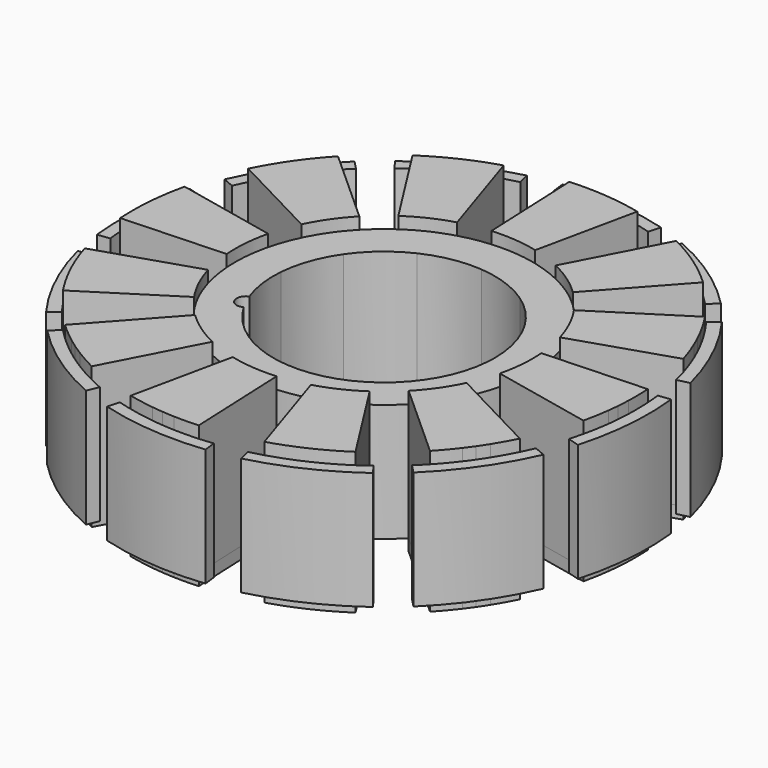
from build123d import *

# Parameters (mm, degrees)
F1_DEPTH      = 5
F2_START      = 5
F2_DEPTH      = 0.5
F3_DEPTH      = 0.5
F4_DEPTH      = 5.5
F4_DEPTH_BACK = 0.5


with BuildPart() as f1:
    # F0 (on Top) → F1 (new body)
    with BuildSketch(Plane.XY):
        with BuildLine():
            Line((3.2158227292, -10.5816797987), (3.0944916155, -10.2076735013))
            ThreePointArc((3.0944916155, -10.2076735013), (2.806845085, -10.2904857677), (2.5169881004, -10.365194044))
            Line((2.5169881004, -10.365194044), (2.6404053121, -10.8734377448))
            ThreePointArc((2.6404053121, -10.8734377448), (4.7631180811, -10.111818259), (6.7021189216, -8.9601892035))
            Line((6.7021189216, -8.9601892035), (6.3888500361, -8.5413741215))
            ThreePointArc((6.3888500361, -8.5413741215), (6.1466771163, -8.7172723426), (5.899664116, -8.8863063185))
            Line((5.899664116, -8.8863063185), (6.1107333051, -9.2180476058))
            Line((6.1107333051, -9.2180476058), (4.6632780172, -9.8998637022))
            Line((4.6632780172, -9.8998637022), (3.2158227292, -10.5816797987))
        make_face()
        with BuildLine():
            ThreePointArc((5.899664116, -8.8863063185), (5.459002884, -9.1636108702), (5.0053347518, -9.4190817328))
            ThreePointArc((5.0053347518, -9.4190817328), (4.7767240343, -9.5370532224), (4.5453347518, -9.6494771185))
            Line((4.5453347518, -9.6494771185), (4.6632780172, -9.8998637022))
            Line((4.6632780172, -9.8998637022), (6.1107333051, -9.2180476058))
            Line((6.1107333051, -9.2180476058), (5.899664116, -8.8863063185))
        make_face()
        with BuildLine():
            ThreePointArc((4.5453347518, -9.6494771185), (4.3362062249, -9.7452445963), (4.1250612878, -9.8364803684))
            ThreePointArc((4.1250612878, -9.8364803684), (3.6145445241, -10.0353148705), (3.0944916155, -10.2076735013))
            Line((3.0944916155, -10.2076735013), (3.2158227292, -10.5816797987))
            Line((3.2158227292, -10.5816797987), (4.6632780172, -9.8998637022))
            Line((4.6632780172, -9.8998637022), (4.5453347518, -9.6494771185))
        make_face()
        with BuildLine():
            Line((-2.5058557218, -10.771914885), (-2.4239283998, -10.3873503734))
            ThreePointArc((-2.4239283998, -10.3873503734), (-2.7144437358, -10.3152446346), (-3.002821386, -10.2350154074))
            Line((-3.002821386, -10.2350154074), (-3.1500607958, -10.7368759695))
            ThreePointArc((-3.1500607958, -10.7368759695), (-0.93092787, -11.1386505313), (1.3241106436, -11.1108109337))
            Line((1.3241106436, -11.1108109337), (1.2622193715, -10.5914719905))
            ThreePointArc((1.2622193715, -10.5914719905), (0.9645423602, -10.6227178585), (0.666105839, -10.6455990756))
            Line((0.666105839, -10.6455990756), (0.6830264751, -11.0384300524))
            Line((0.6830264751, -11.0384300524), (-0.9114146233, -10.9051724687))
            Line((-0.9114146233, -10.9051724687), (-2.5058557218, -10.771914885))
        make_face()
        with BuildLine():
            ThreePointArc((-0.3747938169, -10.6598314368), (-0.6317622506, -10.647692385), (-0.8883631955, -10.6293596938))
            ThreePointArc((-0.8883631955, -10.6293596938), (-1.1173575513, -10.6077324989), (-1.3458323168, -10.5811725268))
            ThreePointArc((-1.3458323168, -10.5811725268), (-1.8873700543, -10.4981098749), (-2.4239283998, -10.3873503734))
            Line((-2.4239283998, -10.3873503734), (-2.5058557218, -10.771914885))
            Line((-2.5058557218, -10.771914885), (-0.9114146233, -10.9051724687))
            Line((-0.9114146233, -10.9051724687), (0.6830264751, -11.0384300524))
            Line((0.6830264751, -11.0384300524), (0.666105839, -10.6455990756))
            ThreePointArc((0.666105839, -10.6455990756), (0.1458297418, -10.6654212459), (-0.3747938169, -10.6598314368))
        make_face()
        with BuildLine():
            Line((-7.5560921558, -8.0758240769), (-7.2928587579, -7.7837451014))
            ThreePointArc((-7.2928587579, -7.7837451014), (-7.5083995497, -7.5760420319), (-7.718027307, -7.362372658))
            Line((-7.718027307, -7.362372658), (-8.0964706574, -7.7233769489))
            ThreePointArc((-8.0964706574, -7.7233769489), (-6.3755324502, -9.180890389), (-4.4086920121, -10.2842998471))
            Line((-4.4086920121, -10.2842998471), (-4.2026219544, -9.803593493))
            ThreePointArc((-4.2026219544, -9.803593493), (-4.4760407423, -9.6818147028), (-4.7459349596, -9.5524121574))
            Line((-4.7459349596, -9.5524121574), (-4.9276967473, -9.9010740809))
            Line((-4.9276967473, -9.9010740809), (-6.2418944516, -8.9884490789))
            Line((-6.2418944516, -8.9884490789), (-7.5560921558, -8.0758240769))
        make_face()
        with BuildLine():
            ThreePointArc((-5.654496685, -9.0442879159), (-5.8709683506, -8.9052909718), (-6.084024942, -8.761113923))
            ThreePointArc((-6.084024942, -8.761113923), (-6.271526274, -8.627887045), (-6.456111239, -8.4906480516))
            ThreePointArc((-6.456111239, -8.4906480516), (-6.8835653508, -8.1479448162), (-7.2928587579, -7.7837451014))
            Line((-7.2928587579, -7.7837451014), (-7.5560921558, -8.0758240769))
            Line((-7.5560921558, -8.0758240769), (-6.2418944516, -8.9884490789))
            Line((-6.2418944516, -8.9884490789), (-4.9276967473, -9.9010740809))
            Line((-4.9276967473, -9.9010740809), (-4.7459349596, -9.5524121574))
            ThreePointArc((-4.7459349596, -9.5524121574), (-5.206418362, -9.3094406119), (-5.654496685, -9.0442879159))
        make_face()
        with BuildLine():
            Line((-10.5816797987, -3.2158227292), (-10.2076735013, -3.0944916155))
            ThreePointArc((-10.2076735013, -3.0944916155), (-10.2904857677, -2.806845085), (-10.365194044, -2.5169881004))
            Line((-10.365194044, -2.5169881004), (-10.8734377448, -2.6404053121))
            ThreePointArc((-10.8734377448, -2.6404053121), (-10.111818259, -4.7631180811), (-8.9601892035, -6.7021189216))
            Line((-8.9601892035, -6.7021189216), (-8.5413741215, -6.3888500361))
            ThreePointArc((-8.5413741215, -6.3888500361), (-8.7172723426, -6.1466771163), (-8.8863063185, -5.899664116))
            Line((-8.8863063185, -5.899664116), (-9.2180476058, -6.1107333051))
            Line((-9.2180476058, -6.1107333051), (-9.8998637022, -4.6632780172))
            Line((-9.8998637022, -4.6632780172), (-10.5816797987, -3.2158227292))
        make_face()
        with BuildLine():
            ThreePointArc((-9.4190817328, -5.0053347518), (-9.5370532224, -4.7767240343), (-9.6494771185, -4.5453347518))
            ThreePointArc((-9.6494771185, -4.5453347518), (-9.7452445963, -4.3362062249), (-9.8364803684, -4.1250612878))
            ThreePointArc((-9.8364803684, -4.1250612878), (-10.0353148705, -3.6145445241), (-10.2076735013, -3.0944916155))
            Line((-10.2076735013, -3.0944916155), (-10.5816797987, -3.2158227292))
            Line((-10.5816797987, -3.2158227292), (-9.8998637022, -4.6632780172))
            Line((-9.8998637022, -4.6632780172), (-9.2180476058, -6.1107333051))
            Line((-9.2180476058, -6.1107333051), (-8.8863063185, -5.899664116))
            ThreePointArc((-8.8863063185, -5.899664116), (-9.1636108702, -5.459002884), (-9.4190817328, -5.0053347518))
        make_face()
        with BuildLine():
            Line((-10.771914885, 2.5058557218), (-10.3873503734, 2.4239283998))
            ThreePointArc((-10.3873503734, 2.4239283998), (-10.3152446346, 2.7144437358), (-10.2350154074, 3.002821386))
            Line((-10.2350154074, 3.002821386), (-10.7368759695, 3.1500607958))
            ThreePointArc((-10.7368759695, 3.1500607958), (-11.1386505313, 0.93092787), (-11.1108109337, -1.3241106436))
            Line((-11.1108109337, -1.3241106436), (-10.5914719905, -1.2622193715))
            ThreePointArc((-10.5914719905, -1.2622193715), (-10.6227178585, -0.9645423602), (-10.6455990756, -0.666105839))
            Line((-10.6455990756, -0.666105839), (-11.0384300524, -0.6830264751))
            Line((-11.0384300524, -0.6830264751), (-10.9051724687, 0.9114146233))
            Line((-10.9051724687, 0.9114146233), (-10.771914885, 2.5058557218))
        make_face()
        with BuildLine():
            ThreePointArc((-10.6598314368, 0.3747938169), (-10.647692385, 0.6317622506), (-10.6293596938, 0.8883631955))
            ThreePointArc((-10.6293596938, 0.8883631955), (-10.6077324989, 1.1173575513), (-10.5811725268, 1.3458323168))
            ThreePointArc((-10.5811725268, 1.3458323168), (-10.4981098749, 1.8873700543), (-10.3873503734, 2.4239283998))
            Line((-10.3873503734, 2.4239283998), (-10.771914885, 2.5058557218))
            Line((-10.771914885, 2.5058557218), (-10.9051724687, 0.9114146233))
            Line((-10.9051724687, 0.9114146233), (-11.0384300524, -0.6830264751))
            Line((-11.0384300524, -0.6830264751), (-10.6455990756, -0.666105839))
            ThreePointArc((-10.6455990756, -0.666105839), (-10.6654212459, -0.1458297418), (-10.6598314368, 0.3747938169))
        make_face()
        with BuildLine():
            Line((8.0758240769, -7.5560921558), (7.7837451014, -7.2928587579))
            ThreePointArc((7.7837451014, -7.2928587579), (7.5760420319, -7.5083995497), (7.362372658, -7.718027307))
            Line((7.362372658, -7.718027307), (7.7233769489, -8.0964706574))
            ThreePointArc((7.7233769489, -8.0964706574), (9.180890389, -6.3755324502), (10.2842998471, -4.4086920121))
            Line((10.2842998471, -4.4086920121), (9.803593493, -4.2026219544))
            ThreePointArc((9.803593493, -4.2026219544), (9.6818147028, -4.4760407423), (9.5524121574, -4.7459349596))
            Line((9.5524121574, -4.7459349596), (9.9010740809, -4.9276967473))
            Line((9.9010740809, -4.9276967473), (8.9884490789, -6.2418944516))
            Line((8.9884490789, -6.2418944516), (8.0758240769, -7.5560921558))
        make_face()
        with BuildLine():
            ThreePointArc((9.0442879159, -5.654496685), (8.9052909718, -5.8709683506), (8.761113923, -6.084024942))
            ThreePointArc((8.761113923, -6.084024942), (8.627887045, -6.271526274), (8.4906480516, -6.456111239))
            ThreePointArc((8.4906480516, -6.456111239), (8.1479448162, -6.8835653508), (7.7837451014, -7.2928587579))
            Line((7.7837451014, -7.2928587579), (8.0758240769, -7.5560921558))
            Line((8.0758240769, -7.5560921558), (8.9884490789, -6.2418944516))
            Line((8.9884490789, -6.2418944516), (9.9010740809, -4.9276967473))
            Line((9.9010740809, -4.9276967473), (9.5524121574, -4.7459349596))
            ThreePointArc((9.5524121574, -4.7459349596), (9.3094406119, -5.206418362), (9.0442879159, -5.654496685))
        make_face()
        with BuildLine():
            Line((10.771914885, -2.5058557218), (10.3873503734, -2.4239283998))
            ThreePointArc((10.3873503734, -2.4239283998), (10.3152446346, -2.7144437358), (10.2350154074, -3.002821386))
            Line((10.2350154074, -3.002821386), (10.7368759695, -3.1500607958))
            ThreePointArc((10.7368759695, -3.1500607958), (11.1386505313, -0.93092787), (11.1108109337, 1.3241106436))
            Line((11.1108109337, 1.3241106436), (10.5914719905, 1.2622193715))
            ThreePointArc((10.5914719905, 1.2622193715), (10.6227178585, 0.9645423602), (10.6455990756, 0.666105839))
            Line((10.6455990756, 0.666105839), (11.0384300524, 0.6830264751))
            Line((11.0384300524, 0.6830264751), (10.9051724687, -0.9114146233))
            Line((10.9051724687, -0.9114146233), (10.771914885, -2.5058557218))
        make_face()
        with BuildLine():
            ThreePointArc((10.6598314368, -0.3747938169), (10.647692385, -0.6317622506), (10.6293596938, -0.8883631955))
            ThreePointArc((10.6293596938, -0.8883631955), (10.6077324989, -1.1173575513), (10.5811725268, -1.3458323168))
            ThreePointArc((10.5811725268, -1.3458323168), (10.4981098749, -1.8873700543), (10.3873503734, -2.4239283998))
            Line((10.3873503734, -2.4239283998), (10.771914885, -2.5058557218))
            Line((10.771914885, -2.5058557218), (10.9051724687, -0.9114146233))
            Line((10.9051724687, -0.9114146233), (11.0384300524, 0.6830264751))
            Line((11.0384300524, 0.6830264751), (10.6455990756, 0.666105839))
            ThreePointArc((10.6455990756, 0.666105839), (10.6654212459, 0.1458297418), (10.6598314368, -0.3747938169))
        make_face()
        with BuildLine():
            Line((10.5816797987, 3.2158227292), (10.2076735013, 3.0944916155))
            ThreePointArc((10.2076735013, 3.0944916155), (10.2904857677, 2.806845085), (10.365194044, 2.5169881004))
            Line((10.365194044, 2.5169881004), (10.8734377448, 2.6404053121))
            ThreePointArc((10.8734377448, 2.6404053121), (10.111818259, 4.7631180811), (8.9601892035, 6.7021189216))
            Line((8.9601892035, 6.7021189216), (8.5413741215, 6.3888500361))
            ThreePointArc((8.5413741215, 6.3888500361), (8.7172723426, 6.1466771163), (8.8863063185, 5.899664116))
            Line((8.8863063185, 5.899664116), (9.2180476058, 6.1107333051))
            Line((9.2180476058, 6.1107333051), (9.8998637022, 4.6632780172))
            Line((9.8998637022, 4.6632780172), (10.5816797987, 3.2158227292))
        make_face()
        with BuildLine():
            ThreePointArc((9.4190817328, 5.0053347518), (9.5370532224, 4.7767240343), (9.6494771185, 4.5453347518))
            ThreePointArc((9.6494771185, 4.5453347518), (9.7452445963, 4.3362062249), (9.8364803684, 4.1250612878))
            ThreePointArc((9.8364803684, 4.1250612878), (10.0353148705, 3.6145445241), (10.2076735013, 3.0944916155))
            Line((10.2076735013, 3.0944916155), (10.5816797987, 3.2158227292))
            Line((10.5816797987, 3.2158227292), (9.8998637022, 4.6632780172))
            Line((9.8998637022, 4.6632780172), (9.2180476058, 6.1107333051))
            Line((9.2180476058, 6.1107333051), (8.8863063185, 5.899664116))
            ThreePointArc((8.8863063185, 5.899664116), (9.1636108702, 5.459002884), (9.4190817328, 5.0053347518))
        make_face()
        with BuildLine():
            Line((7.5560921558, 8.0758240769), (7.2928587579, 7.7837451014))
            ThreePointArc((7.2928587579, 7.7837451014), (7.5083995497, 7.5760420319), (7.718027307, 7.362372658))
            Line((7.718027307, 7.362372658), (8.0964706574, 7.7233769489))
            ThreePointArc((8.0964706574, 7.7233769489), (6.3755324502, 9.180890389), (4.4086920121, 10.2842998471))
            Line((4.4086920121, 10.2842998471), (4.2026219544, 9.803593493))
            ThreePointArc((4.2026219544, 9.803593493), (4.4760407423, 9.6818147028), (4.7459349596, 9.5524121574))
            Line((4.7459349596, 9.5524121574), (4.9276967473, 9.9010740809))
            Line((4.9276967473, 9.9010740809), (6.2418944516, 8.9884490789))
            Line((6.2418944516, 8.9884490789), (7.5560921558, 8.0758240769))
        make_face()
        with BuildLine():
            ThreePointArc((5.654496685, 9.0442879159), (5.8709683506, 8.9052909718), (6.084024942, 8.761113923))
            ThreePointArc((6.084024942, 8.761113923), (6.271526274, 8.627887045), (6.456111239, 8.4906480516))
            ThreePointArc((6.456111239, 8.4906480516), (6.8835653508, 8.1479448162), (7.2928587579, 7.7837451014))
            Line((7.2928587579, 7.7837451014), (7.5560921558, 8.0758240769))
            Line((7.5560921558, 8.0758240769), (6.2418944516, 8.9884490789))
            Line((6.2418944516, 8.9884490789), (4.9276967473, 9.9010740809))
            Line((4.9276967473, 9.9010740809), (4.7459349596, 9.5524121574))
            ThreePointArc((4.7459349596, 9.5524121574), (5.206418362, 9.3094406119), (5.654496685, 9.0442879159))
        make_face()
        with BuildLine():
            Line((2.5058557218, 10.771914885), (2.4239283998, 10.3873503734))
            ThreePointArc((2.4239283998, 10.3873503734), (2.7144437358, 10.3152446346), (3.002821386, 10.2350154074))
            Line((3.002821386, 10.2350154074), (3.1500607958, 10.7368759695))
            ThreePointArc((3.1500607958, 10.7368759695), (0.93092787, 11.1386505313), (-1.3241106436, 11.1108109337))
            Line((-1.3241106436, 11.1108109337), (-1.2622193715, 10.5914719905))
            ThreePointArc((-1.2622193715, 10.5914719905), (-0.9645423602, 10.6227178585), (-0.666105839, 10.6455990756))
            Line((-0.666105839, 10.6455990756), (-0.6830264751, 11.0384300524))
            Line((-0.6830264751, 11.0384300524), (0.9114146233, 10.9051724687))
            Line((0.9114146233, 10.9051724687), (2.5058557218, 10.771914885))
        make_face()
        with BuildLine():
            ThreePointArc((0.3747938169, 10.6598314368), (0.6317622506, 10.647692385), (0.8883631955, 10.6293596938))
            ThreePointArc((0.8883631955, 10.6293596938), (1.1173575513, 10.6077324989), (1.3458323168, 10.5811725268))
            ThreePointArc((1.3458323168, 10.5811725268), (1.8873700543, 10.4981098749), (2.4239283998, 10.3873503734))
            Line((2.4239283998, 10.3873503734), (2.5058557218, 10.771914885))
            Line((2.5058557218, 10.771914885), (0.9114146233, 10.9051724687))
            Line((0.9114146233, 10.9051724687), (-0.6830264751, 11.0384300524))
            Line((-0.6830264751, 11.0384300524), (-0.666105839, 10.6455990756))
            ThreePointArc((-0.666105839, 10.6455990756), (-0.1458297418, 10.6654212459), (0.3747938169, 10.6598314368))
        make_face()
        with BuildLine():
            Line((-3.2158227292, 10.5816797987), (-3.0944916155, 10.2076735013))
            ThreePointArc((-3.0944916155, 10.2076735013), (-2.806845085, 10.2904857677), (-2.5169881004, 10.365194044))
            Line((-2.5169881004, 10.365194044), (-2.6404053121, 10.8734377448))
            ThreePointArc((-2.6404053121, 10.8734377448), (-4.7631180811, 10.111818259), (-6.7021189216, 8.9601892035))
            Line((-6.7021189216, 8.9601892035), (-6.3888500361, 8.5413741215))
            ThreePointArc((-6.3888500361, 8.5413741215), (-6.1466771163, 8.7172723426), (-5.899664116, 8.8863063185))
            Line((-5.899664116, 8.8863063185), (-6.1107333051, 9.2180476058))
            Line((-6.1107333051, 9.2180476058), (-4.6632780172, 9.8998637022))
            Line((-4.6632780172, 9.8998637022), (-3.2158227292, 10.5816797987))
        make_face()
        with BuildLine():
            ThreePointArc((-5.0053347518, 9.4190817328), (-4.7767240343, 9.5370532224), (-4.5453347518, 9.6494771185))
            ThreePointArc((-4.5453347518, 9.6494771185), (-4.3362062249, 9.7452445963), (-4.1250612878, 9.8364803684))
            ThreePointArc((-4.1250612878, 9.8364803684), (-3.6145445241, 10.0353148705), (-3.0944916155, 10.2076735013))
            Line((-3.0944916155, 10.2076735013), (-3.2158227292, 10.5816797987))
            Line((-3.2158227292, 10.5816797987), (-4.6632780172, 9.8998637022))
            Line((-4.6632780172, 9.8998637022), (-6.1107333051, 9.2180476058))
            Line((-6.1107333051, 9.2180476058), (-5.899664116, 8.8863063185))
            ThreePointArc((-5.899664116, 8.8863063185), (-5.459002884, 9.1636108702), (-5.0053347518, 9.4190817328))
        make_face()
        with BuildLine():
            Line((-8.0758240769, 7.5560921558), (-7.7837451014, 7.2928587579))
            ThreePointArc((-7.7837451014, 7.2928587579), (-7.5760420319, 7.5083995497), (-7.362372658, 7.718027307))
            Line((-7.362372658, 7.718027307), (-7.7233769489, 8.0964706574))
            ThreePointArc((-7.7233769489, 8.0964706574), (-9.180890389, 6.3755324502), (-10.2842998471, 4.4086920121))
            Line((-10.2842998471, 4.4086920121), (-9.803593493, 4.2026219544))
            ThreePointArc((-9.803593493, 4.2026219544), (-9.6818147028, 4.4760407423), (-9.5524121574, 4.7459349596))
            Line((-9.5524121574, 4.7459349596), (-9.9010740809, 4.9276967473))
            Line((-9.9010740809, 4.9276967473), (-8.9884490789, 6.2418944516))
            Line((-8.9884490789, 6.2418944516), (-8.0758240769, 7.5560921558))
        make_face()
        with BuildLine():
            ThreePointArc((-9.0442879159, 5.654496685), (-8.9052909718, 5.8709683506), (-8.761113923, 6.084024942))
            ThreePointArc((-8.761113923, 6.084024942), (-8.627887045, 6.271526274), (-8.4906480516, 6.456111239))
            ThreePointArc((-8.4906480516, 6.456111239), (-8.1479448162, 6.8835653508), (-7.7837451014, 7.2928587579))
            Line((-7.7837451014, 7.2928587579), (-8.0758240769, 7.5560921558))
            Line((-8.0758240769, 7.5560921558), (-8.9884490789, 6.2418944516))
            Line((-8.9884490789, 6.2418944516), (-9.9010740809, 4.9276967473))
            Line((-9.9010740809, 4.9276967473), (-9.5524121574, 4.7459349596))
            ThreePointArc((-9.5524121574, 4.7459349596), (-9.3094406119, 5.206418362), (-9.0442879159, 5.654496685))
        make_face()
        with BuildLine():
            ThreePointArc((-4.6784977785, 0.391011816), (-4.4178805277, 1.588572739), (-3.8561920198, 2.6778750551))
            Line((-3.8561920198, 2.6778750551), (-4.5953452184, 3.1911689736))
            Line((-4.5953452184, 3.1911689736), (-4.8571806853, 2.8129597878))
            Line((-4.8571806853, 2.8129597878), (-5.1190161522, 2.4347506019))
            Line((-5.1190161522, 2.4347506019), (-5.6824068137, 2.7284531456))
            ThreePointArc((-5.6824068137, 2.7284531456), (-5.9317597041, 2.1327049906), (-6.1188464962, 1.5145696814))
            Line((-6.1188464962, 1.5145696814), (-5.4986734774, 1.3824485078))
            Line((-5.4986734774, 1.3824485078), (-5.5369718313, 0.9242046488))
            Line((-5.5369718313, 0.9242046488), (-5.5752701851, 0.4659607897))
            Line((-5.5752701851, 0.4659607897), (-4.6784977785, 0.391011816))
        make_face()
        with BuildLine():
            Line((-3.1911689736, -4.5953452184), (-2.6778750551, -3.8561920198))
            ThreePointArc((-2.6778750551, -3.8561920198), (-3.4532961184, -3.1805624695), (-4.0629943776, -2.3522985337))
            ThreePointArc((-4.0629943776, -2.3522985337), (-4.3736064249, -2.3769621785), (-4.6063536791, -2.1697983424))
            Line((-4.6063536791, -2.1697983424), (-5.0613060081, -2.3841012115))
            Line((-5.0613060081, -2.3841012115), (-4.8646849787, -2.7999619704))
            Line((-4.8646849787, -2.7999619704), (-4.6680639492, -3.2158227292))
            Line((-4.6680639492, -3.2158227292), (-5.204113144, -3.5568820825))
            ThreePointArc((-5.204113144, -3.5568820825), (-4.8128565527, -4.0707020976), (-4.371079068, -4.5417916669))
            Line((-4.371079068, -4.5417916669), (-3.9465722659, -4.0707666646))
            Line((-3.9465722659, -4.0707666646), (-3.5688706198, -4.3330559415))
            Line((-3.5688706198, -4.3330559415), (-3.1911689736, -4.5953452184))
        make_face()
        with BuildLine():
            ThreePointArc((-0.391011816, -4.6784977785), (-1.588572739, -4.4178805277), (-2.6778750551, -3.8561920198))
            Line((-2.6778750551, -3.8561920198), (-3.1911689736, -4.5953452184))
            Line((-3.1911689736, -4.5953452184), (-2.8129597878, -4.8571806853))
            Line((-2.8129597878, -4.8571806853), (-2.4347506019, -5.1190161522))
            Line((-2.4347506019, -5.1190161522), (-2.7284531456, -5.6824068137))
            ThreePointArc((-2.7284531456, -5.6824068137), (-2.1327049906, -5.9317597041), (-1.5145696814, -6.1188464962))
            Line((-1.5145696814, -6.1188464962), (-1.3824485078, -5.4986734774))
            Line((-1.3824485078, -5.4986734774), (-0.9242046488, -5.5369718313))
            Line((-0.9242046488, -5.5369718313), (-0.4659607897, -5.5752701851))
            Line((-0.4659607897, -5.5752701851), (-0.391011816, -4.6784977785))
        make_face()
        with BuildLine():
            Line((2.3841012115, -5.0613060081), (2.0006227234, -4.2472038357))
            ThreePointArc((2.0006227234, -4.2472038357), (0.8331959161, -4.6202831373), (-0.391011816, -4.6784977785))
            Line((-0.391011816, -4.6784977785), (-0.4659607897, -5.5752701851))
            Line((-0.4659607897, -5.5752701851), (-0.0075042934, -5.6129217581))
            Line((-0.0075042934, -5.6129217581), (0.450952203, -5.6505733311))
            Line((0.450952203, -5.6505733311), (0.4782936697, -6.2853352281))
            ThreePointArc((0.4782936697, -6.2853352281), (1.1189031514, -6.2034070882), (1.7477674282, -6.0563613483))
            Line((1.7477674282, -6.0563613483), (1.5521012115, -5.4532151725))
            Line((1.5521012115, -5.4532151725), (1.9681012115, -5.2572605903))
            Line((1.9681012115, -5.2572605903), (2.3841012115, -5.0613060081))
        make_face()
        with BuildLine():
            Line((4.5953452184, -3.1911689736), (3.8561920198, -2.6778750551))
            ThreePointArc((3.8561920198, -2.6778750551), (3.0317103984, -3.5846846116), (2.0006227234, -4.2472038357))
            Line((2.0006227234, -4.2472038357), (2.3841012115, -5.0613060081))
            Line((2.3841012115, -5.0613060081), (2.7999619704, -4.8646849787))
            Line((2.7999619704, -4.8646849787), (3.2158227292, -4.6680639492))
            Line((3.2158227292, -4.6680639492), (3.5568820825, -5.204113144))
            ThreePointArc((3.5568820825, -5.204113144), (4.0707020976, -4.8128565527), (4.5417916669, -4.371079068))
            Line((4.5417916669, -4.371079068), (4.0707666646, -3.9465722659))
            Line((4.0707666646, -3.9465722659), (4.3330559415, -3.5688706198))
            Line((4.3330559415, -3.5688706198), (4.5953452184, -3.1911689736))
        make_face()
        with BuildLine():
            Line((5.5752701851, -0.4659607897), (4.6784977785, -0.391011816))
            ThreePointArc((4.6784977785, -0.391011816), (4.4178805277, -1.588572739), (3.8561920198, -2.6778750551))
            Line((3.8561920198, -2.6778750551), (4.5953452184, -3.1911689736))
            Line((4.5953452184, -3.1911689736), (4.8571806853, -2.8129597878))
            Line((4.8571806853, -2.8129597878), (5.1190161522, -2.4347506019))
            Line((5.1190161522, -2.4347506019), (5.6824068137, -2.7284531456))
            ThreePointArc((5.6824068137, -2.7284531456), (5.9317597041, -2.1327049906), (6.1188464962, -1.5145696814))
            Line((6.1188464962, -1.5145696814), (5.4986734774, -1.3824485078))
            Line((5.4986734774, -1.3824485078), (5.5369718313, -0.9242046488))
            Line((5.5369718313, -0.9242046488), (5.5752701851, -0.4659607897))
        make_face()
        with BuildLine():
            Line((5.0613060081, 2.3841012115), (4.2472038357, 2.0006227234))
            ThreePointArc((4.2472038357, 2.0006227234), (4.5815413655, 1.0250416674), (4.6948090168, 0))
            ThreePointArc((4.6948090168, 0), (4.6907294347, -0.1956759418), (4.6784977785, -0.391011816))
            Line((4.6784977785, -0.391011816), (5.5752701851, -0.4659607897))
            Line((5.5752701851, -0.4659607897), (5.6129217581, -0.0075042934))
            Line((5.6129217581, -0.0075042934), (5.6505733311, 0.450952203))
            Line((5.6505733311, 0.450952203), (6.2853352281, 0.4782936697))
            ThreePointArc((6.2853352281, 0.4782936697), (6.2034070882, 1.1189031514), (6.0563613483, 1.7477674282))
            Line((6.0563613483, 1.7477674282), (5.4532151725, 1.5521012115))
            Line((5.4532151725, 1.5521012115), (5.2572605903, 1.9681012115))
            Line((5.2572605903, 1.9681012115), (5.0613060081, 2.3841012115))
        make_face()
        with BuildLine():
            ThreePointArc((2.6778750551, 3.8561920198), (3.5846846116, 3.0317103984), (4.2472038357, 2.0006227234))
            Line((4.2472038357, 2.0006227234), (5.0613060081, 2.3841012115))
            Line((5.0613060081, 2.3841012115), (4.8646849787, 2.7999619704))
            Line((4.8646849787, 2.7999619704), (4.6680639492, 3.2158227292))
            Line((4.6680639492, 3.2158227292), (5.204113144, 3.5568820825))
            ThreePointArc((5.204113144, 3.5568820825), (4.8128565527, 4.0707020976), (4.371079068, 4.5417916669))
            Line((4.371079068, 4.5417916669), (3.9465722659, 4.0707666646))
            Line((3.9465722659, 4.0707666646), (3.5688706198, 4.3330559415))
            Line((3.5688706198, 4.3330559415), (3.1911689736, 4.5953452184))
            Line((3.1911689736, 4.5953452184), (2.6778750551, 3.8561920198))
        make_face()
        with BuildLine():
            ThreePointArc((0.391011816, 4.6784977785), (1.588572739, 4.4178805277), (2.6778750551, 3.8561920198))
            Line((2.6778750551, 3.8561920198), (3.1911689736, 4.5953452184))
            Line((3.1911689736, 4.5953452184), (2.8129597878, 4.8571806853))
            Line((2.8129597878, 4.8571806853), (2.4347506019, 5.1190161522))
            Line((2.4347506019, 5.1190161522), (2.7284531456, 5.6824068137))
            ThreePointArc((2.7284531456, 5.6824068137), (2.1327049906, 5.9317597041), (1.5145696814, 6.1188464962))
            Line((1.5145696814, 6.1188464962), (1.3824485078, 5.4986734774))
            Line((1.3824485078, 5.4986734774), (0.9242046488, 5.5369718313))
            Line((0.9242046488, 5.5369718313), (0.4659607897, 5.5752701851))
            Line((0.4659607897, 5.5752701851), (0.391011816, 4.6784977785))
        make_face()
        with BuildLine():
            ThreePointArc((-2.0006227234, 4.2472038357), (-0.8331959161, 4.6202831373), (0.391011816, 4.6784977785))
            Line((0.391011816, 4.6784977785), (0.4659607897, 5.5752701851))
            Line((0.4659607897, 5.5752701851), (0.0075042934, 5.6129217581))
            Line((0.0075042934, 5.6129217581), (-0.450952203, 5.6505733311))
            Line((-0.450952203, 5.6505733311), (-0.4782936697, 6.2853352281))
            ThreePointArc((-0.4782936697, 6.2853352281), (-1.1189031514, 6.2034070882), (-1.7477674282, 6.0563613483))
            Line((-1.7477674282, 6.0563613483), (-1.5521012115, 5.4532151725))
            Line((-1.5521012115, 5.4532151725), (-1.9681012115, 5.2572605903))
            Line((-1.9681012115, 5.2572605903), (-2.3841012115, 5.0613060081))
            Line((-2.3841012115, 5.0613060081), (-2.0006227234, 4.2472038357))
        make_face()
        with BuildLine():
            ThreePointArc((-3.8561920198, 2.6778750551), (-3.0317103984, 3.5846846116), (-2.0006227234, 4.2472038357))
            Line((-2.0006227234, 4.2472038357), (-2.3841012115, 5.0613060081))
            Line((-2.3841012115, 5.0613060081), (-2.7999619704, 4.8646849787))
            Line((-2.7999619704, 4.8646849787), (-3.2158227292, 4.6680639492))
            Line((-3.2158227292, 4.6680639492), (-3.5568820825, 5.204113144))
            ThreePointArc((-3.5568820825, 5.204113144), (-4.0707020976, 4.8128565527), (-4.5417916669, 4.371079068))
            Line((-4.5417916669, 4.371079068), (-4.0707666646, 3.9465722659))
            Line((-4.0707666646, 3.9465722659), (-4.3330559415, 3.5688706198))
            Line((-4.3330559415, 3.5688706198), (-4.5953452184, 3.1911689736))
            Line((-4.5953452184, 3.1911689736), (-3.8561920198, 2.6778750551))
        make_face()
        with BuildLine():
            ThreePointArc((-4.4010430515, -1.6346411724), (-4.6513796801, -0.6371018564), (-4.6784977785, 0.391011816))
            Line((-4.6784977785, 0.391011816), (-5.5752701851, 0.4659607897))
            Line((-5.5752701851, 0.4659607897), (-5.6129217581, 0.0075042934))
            Line((-5.6129217581, 0.0075042934), (-5.6505733311, -0.450952203))
            Line((-5.6505733311, -0.450952203), (-6.2853352281, -0.4782936697))
            ThreePointArc((-6.2853352281, -0.4782936697), (-6.2034070882, -1.1189031514), (-6.0563613483, -1.7477674282))
            Line((-6.0563613483, -1.7477674282), (-5.4532151725, -1.5521012115))
            Line((-5.4532151725, -1.5521012115), (-5.2572605903, -1.9681012115))
            Line((-5.2572605903, -1.9681012115), (-5.0613060081, -2.3841012115))
            Line((-5.0613060081, -2.3841012115), (-4.6063536791, -2.1697983424))
            ThreePointArc((-4.6063536791, -2.1697983424), (-4.6178623616, -1.8584212566), (-4.4010430515, -1.6346411724))
        make_face()
        with BuildLine():
            Line((2.8841012115, -6.1227764658), (2.6861454459, -5.7025280716))
            ThreePointArc((2.6861454459, -5.7025280716), (2.4762136655, -5.7967723474), (2.2629818624, -5.8832913284))
            Line((2.2629818624, -5.8832913284), (4.1250612878, -9.8364803684))
            ThreePointArc((4.1250612878, -9.8364803684), (4.3362062249, -9.7452445963), (4.5453347518, -9.6494771185))
            Line((4.5453347518, -9.6494771185), (2.8841012115, -6.1227764658))
        make_face()
        with BuildLine():
            ThreePointArc((3.101614921, -5.4876396243), (2.8958740956, -5.5989389161), (2.6861454459, -5.7025280716))
            Line((2.6861454459, -5.7025280716), (2.8841012115, -6.1227764658))
            Line((2.8841012115, -6.1227764658), (4.5453347518, -9.6494771185))
            ThreePointArc((4.5453347518, -9.6494771185), (4.7767240343, -9.5370532224), (5.0053347518, -9.4190817328))
            Line((5.0053347518, -9.4190817328), (3.101614921, -5.4876396243))
        make_face()
        with BuildLine():
            Line((2.2629818624, -5.8832913284), (1.9681012115, -5.2572605903))
            Line((1.9681012115, -5.2572605903), (1.5521012115, -5.4532151725))
            Line((1.5521012115, -5.4532151725), (1.7477674282, -6.0563613483))
            ThreePointArc((1.7477674282, -6.0563613483), (2.0072408365, -5.9753818278), (2.2629818624, -5.8832913284))
        make_face()
        with BuildLine():
            Line((2.6861454459, -5.7025280716), (2.3841012115, -5.0613060081))
            Line((2.3841012115, -5.0613060081), (1.9681012115, -5.2572605903))
            Line((1.9681012115, -5.2572605903), (2.2629818624, -5.8832913284))
            ThreePointArc((2.2629818624, -5.8832913284), (2.4762136655, -5.7967723474), (2.6861454459, -5.7025280716))
        make_face()
        with BuildLine():
            Line((2.7999619704, -4.8646849787), (2.3841012115, -5.0613060081))
            Line((2.3841012115, -5.0613060081), (2.6861454459, -5.7025280716))
            ThreePointArc((2.6861454459, -5.7025280716), (2.8958740956, -5.5989389161), (3.101614921, -5.4876396243))
            Line((3.101614921, -5.4876396243), (2.7999619704, -4.8646849787))
        make_face()
        with BuildLine():
            Line((3.2158227292, -4.6680639492), (2.7999619704, -4.8646849787))
            Line((2.7999619704, -4.8646849787), (3.101614921, -5.4876396243))
            ThreePointArc((3.101614921, -5.4876396243), (3.332265356, -5.3507206395), (3.5568820825, -5.204113144))
            Line((3.5568820825, -5.204113144), (3.2158227292, -4.6680639492))
        make_face()
        with BuildLine():
            ThreePointArc((-0.0577424978, -6.3032427819), (-0.2915689251, -6.2967603834), (-0.5249938414, -6.2816068988))
            Line((-0.5249938414, -6.2816068988), (-0.8883631955, -10.6293596938))
            ThreePointArc((-0.8883631955, -10.6293596938), (-0.6317622506, -10.647692385), (-0.3747938169, -10.6598314368))
            Line((-0.3747938169, -10.6598314368), (-0.0577424978, -6.3032427819))
        make_face()
        with BuildLine():
            Line((-0.8883631955, -10.6293596938), (-0.5249938414, -6.2816068988))
            ThreePointArc((-0.5249938414, -6.2816068988), (-0.7539222342, -6.2582589455), (-0.9818458831, -6.2265706794))
            Line((-0.9818458831, -6.2265706794), (-1.3458323168, -10.5811725268))
            ThreePointArc((-1.3458323168, -10.5811725268), (-1.1173575513, -10.6077324989), (-0.8883631955, -10.6293596938))
        make_face()
        with BuildLine():
            Line((0.450952203, -5.6505733311), (-0.0075042934, -5.6129217581))
            Line((-0.0075042934, -5.6129217581), (-0.0577424978, -6.3032427819))
            ThreePointArc((-0.0577424978, -6.3032427819), (0.2104661307, -6.2999926803), (0.4782936697, -6.2853352281))
            Line((0.4782936697, -6.2853352281), (0.450952203, -5.6505733311))
        make_face()
        with BuildLine():
            Line((-0.9818458831, -6.2265706794), (-0.9242046488, -5.5369718313))
            Line((-0.9242046488, -5.5369718313), (-1.3824485078, -5.4986734774))
            Line((-1.3824485078, -5.4986734774), (-1.5145696814, -6.1188464962))
            ThreePointArc((-1.5145696814, -6.1188464962), (-1.249369358, -6.1784528785), (-0.9818458831, -6.2265706794))
        make_face()
        with BuildLine():
            Line((-0.5249938414, -6.2816068988), (-0.4659607897, -5.5752701851))
            Line((-0.4659607897, -5.5752701851), (-0.9242046488, -5.5369718313))
            Line((-0.9242046488, -5.5369718313), (-0.9818458831, -6.2265706794))
            ThreePointArc((-0.9818458831, -6.2265706794), (-0.7539222342, -6.2582589455), (-0.5249938414, -6.2816068988))
        make_face()
        with BuildLine():
            Line((-0.0075042934, -5.6129217581), (-0.4659607897, -5.5752701851))
            Line((-0.4659607897, -5.5752701851), (-0.5249938414, -6.2816068988))
            ThreePointArc((-0.5249938414, -6.2816068988), (-0.2915689251, -6.2967603834), (-0.0577424978, -6.3032427819))
            Line((-0.0577424978, -6.3032427819), (-0.0075042934, -5.6129217581))
        make_face()
        with BuildLine():
            ThreePointArc((-3.2016278609, -5.4298971265), (-3.4008862878, -5.307369991), (-3.5954614529, -5.1775342302))
            Line((-3.5954614529, -5.1775342302), (-6.084024942, -8.761113923))
            ThreePointArc((-6.084024942, -8.761113923), (-5.8709683506, -8.9052909718), (-5.654496685, -9.0442879159))
            Line((-5.654496685, -9.0442879159), (-3.2016278609, -5.4298971265))
        make_face()
        with BuildLine():
            Line((-2.8129597878, -4.8571806853), (-3.1911689736, -4.5953452184))
            Line((-3.1911689736, -4.5953452184), (-3.5954614529, -5.1775342302))
            ThreePointArc((-3.5954614529, -5.1775342302), (-3.4008862878, -5.307369991), (-3.2016278609, -5.4298971265))
            Line((-3.2016278609, -5.4298971265), (-2.8129597878, -4.8571806853))
        make_face()
        with BuildLine():
            Line((-3.5954614529, -5.1775342302), (-3.1911689736, -4.5953452184))
            Line((-3.1911689736, -4.5953452184), (-3.5688706198, -4.3330559415))
            Line((-3.5688706198, -4.3330559415), (-3.9635888171, -4.9014454453))
            ThreePointArc((-3.9635888171, -4.9014454453), (-3.78204528, -5.0428501132), (-3.5954614529, -5.1775342302))
        make_face()
        with BuildLine():
            Line((-6.084024942, -8.761113923), (-3.5954614529, -5.1775342302))
            ThreePointArc((-3.5954614529, -5.1775342302), (-3.78204528, -5.0428501132), (-3.9635888171, -4.9014454453))
            Line((-3.9635888171, -4.9014454453), (-6.456111239, -8.4906480516))
            ThreePointArc((-6.456111239, -8.4906480516), (-6.271526274, -8.627887045), (-6.084024942, -8.761113923))
        make_face()
        with BuildLine():
            Line((8.761113923, -6.084024942), (5.1775342302, -3.5954614529))
            ThreePointArc((5.1775342302, -3.5954614529), (5.0428501132, -3.78204528), (4.9014454453, -3.9635888171))
            Line((4.9014454453, -3.9635888171), (8.4906480516, -6.456111239))
            ThreePointArc((8.4906480516, -6.456111239), (8.627887045, -6.271526274), (8.761113923, -6.084024942))
        make_face()
        with BuildLine():
            ThreePointArc((5.4298971265, -3.2016278609), (5.307369991, -3.4008862878), (5.1775342302, -3.5954614529))
            Line((5.1775342302, -3.5954614529), (8.761113923, -6.084024942))
            ThreePointArc((8.761113923, -6.084024942), (8.9052909718, -5.8709683506), (9.0442879159, -5.654496685))
            Line((9.0442879159, -5.654496685), (5.4298971265, -3.2016278609))
        make_face()
        with BuildLine():
            Line((4.8571806853, -2.8129597878), (4.5953452184, -3.1911689736))
            Line((4.5953452184, -3.1911689736), (5.1775342302, -3.5954614529))
            ThreePointArc((5.1775342302, -3.5954614529), (5.307369991, -3.4008862878), (5.4298971265, -3.2016278609))
            Line((5.4298971265, -3.2016278609), (4.8571806853, -2.8129597878))
        make_face()
        with BuildLine():
            Line((5.1190161522, -2.4347506019), (4.8571806853, -2.8129597878))
            Line((4.8571806853, -2.8129597878), (5.4298971265, -3.2016278609))
            ThreePointArc((5.4298971265, -3.2016278609), (5.5611867702, -2.9677273243), (5.6824068137, -2.7284531456))
            Line((5.6824068137, -2.7284531456), (5.1190161522, -2.4347506019))
        make_face()
        with BuildLine():
            Line((5.1775342302, -3.5954614529), (4.5953452184, -3.1911689736))
            Line((4.5953452184, -3.1911689736), (4.3330559415, -3.5688706198))
            Line((4.3330559415, -3.5688706198), (4.9014454453, -3.9635888171))
            ThreePointArc((4.9014454453, -3.9635888171), (5.0428501132, -3.78204528), (5.1775342302, -3.5954614529))
        make_face()
        with BuildLine():
            Line((4.9014454453, -3.9635888171), (4.3330559415, -3.5688706198))
            Line((4.3330559415, -3.5688706198), (4.0707666646, -3.9465722659))
            Line((4.0707666646, -3.9465722659), (4.5417916669, -4.371079068))
            ThreePointArc((4.5417916669, -4.371079068), (4.7260124699, -4.1712120419), (4.9014454453, -3.9635888171))
        make_face()
        with BuildLine():
            Line((6.2265706794, -0.9818458831), (5.5369718313, -0.9242046488))
            Line((5.5369718313, -0.9242046488), (5.4986734774, -1.3824485078))
            Line((5.4986734774, -1.3824485078), (6.1188464962, -1.5145696814))
            ThreePointArc((6.1188464962, -1.5145696814), (6.1784528785, -1.249369358), (6.2265706794, -0.9818458831))
        make_face()
        with BuildLine():
            Line((6.2816068988, -0.5249938414), (5.5752701851, -0.4659607897))
            Line((5.5752701851, -0.4659607897), (5.5369718313, -0.9242046488))
            Line((5.5369718313, -0.9242046488), (6.2265706794, -0.9818458831))
            ThreePointArc((6.2265706794, -0.9818458831), (6.2582589455, -0.7539222342), (6.2816068988, -0.5249938414))
        make_face()
        with BuildLine():
            Line((5.6129217581, -0.0075042934), (5.5752701851, -0.4659607897))
            Line((5.5752701851, -0.4659607897), (6.2816068988, -0.5249938414))
            ThreePointArc((6.2816068988, -0.5249938414), (6.2967603834, -0.2915689251), (6.3032427819, -0.0577424978))
            Line((6.3032427819, -0.0577424978), (5.6129217581, -0.0075042934))
        make_face()
        with BuildLine():
            Line((5.6505733311, 0.450952203), (5.6129217581, -0.0075042934))
            Line((5.6129217581, -0.0075042934), (6.3032427819, -0.0577424978))
            ThreePointArc((6.3032427819, -0.0577424978), (6.3034411394, -0.0288715517), (6.303507259, 0))
            ThreePointArc((6.303507259, 0), (6.298962613, 0.2393193772), (6.2853352281, 0.4782936697))
            Line((6.2853352281, 0.4782936697), (5.6505733311, 0.450952203))
        make_face()
        with BuildLine():
            ThreePointArc((6.3032427819, -0.0577424978), (6.2967603834, -0.2915689251), (6.2816068988, -0.5249938414))
            Line((6.2816068988, -0.5249938414), (10.6293596938, -0.8883631955))
            ThreePointArc((10.6293596938, -0.8883631955), (10.647692385, -0.6317622506), (10.6598314368, -0.3747938169))
            Line((10.6598314368, -0.3747938169), (6.3032427819, -0.0577424978))
        make_face()
        with BuildLine():
            Line((10.6293596938, -0.8883631955), (6.2816068988, -0.5249938414))
            ThreePointArc((6.2816068988, -0.5249938414), (6.2582589455, -0.7539222342), (6.2265706794, -0.9818458831))
            Line((6.2265706794, -0.9818458831), (10.5811725268, -1.3458323168))
            ThreePointArc((10.5811725268, -1.3458323168), (10.6077324989, -1.1173575513), (10.6293596938, -0.8883631955))
        make_face()
        with BuildLine():
            ThreePointArc((5.4876396243, 3.101614921), (5.5989389161, 2.8958740956), (5.7025280716, 2.6861454459))
            Line((5.7025280716, 2.6861454459), (9.6494771185, 4.5453347518))
            ThreePointArc((9.6494771185, 4.5453347518), (9.5370532224, 4.7767240343), (9.4190817328, 5.0053347518))
            Line((9.4190817328, 5.0053347518), (5.4876396243, 3.101614921))
        make_face()
        with BuildLine():
            Line((9.6494771185, 4.5453347518), (5.7025280716, 2.6861454459))
            ThreePointArc((5.7025280716, 2.6861454459), (5.7967723474, 2.4762136655), (5.8832913284, 2.2629818624))
            Line((5.8832913284, 2.2629818624), (9.8364803684, 4.1250612878))
            ThreePointArc((9.8364803684, 4.1250612878), (9.7452445963, 4.3362062249), (9.6494771185, 4.5453347518))
        make_face()
        with BuildLine():
            Line((4.8646849787, 2.7999619704), (5.0613060081, 2.3841012115))
            Line((5.0613060081, 2.3841012115), (5.7025280716, 2.6861454459))
            ThreePointArc((5.7025280716, 2.6861454459), (5.5989389161, 2.8958740956), (5.4876396243, 3.101614921))
            Line((5.4876396243, 3.101614921), (4.8646849787, 2.7999619704))
        make_face()
        with BuildLine():
            Line((4.6680639492, 3.2158227292), (4.8646849787, 2.7999619704))
            Line((4.8646849787, 2.7999619704), (5.4876396243, 3.101614921))
            ThreePointArc((5.4876396243, 3.101614921), (5.3507206395, 3.332265356), (5.204113144, 3.5568820825))
            Line((5.204113144, 3.5568820825), (4.6680639492, 3.2158227292))
        make_face()
        with BuildLine():
            Line((5.7025280716, 2.6861454459), (5.0613060081, 2.3841012115))
            Line((5.0613060081, 2.3841012115), (5.2572605903, 1.9681012115))
            Line((5.2572605903, 1.9681012115), (5.8832913284, 2.2629818624))
            ThreePointArc((5.8832913284, 2.2629818624), (5.7967723474, 2.4762136655), (5.7025280716, 2.6861454459))
        make_face()
        with BuildLine():
            Line((5.8832913284, 2.2629818624), (5.2572605903, 1.9681012115))
            Line((5.2572605903, 1.9681012115), (5.4532151725, 1.5521012115))
            Line((5.4532151725, 1.5521012115), (6.0563613483, 1.7477674282))
            ThreePointArc((6.0563613483, 1.7477674282), (5.9753818278, 2.0072408365), (5.8832913284, 2.2629818624))
        make_face()
        with BuildLine():
            ThreePointArc((-5.4876396243, -3.101614921), (-5.5989389161, -2.8958740956), (-5.7025280716, -2.6861454459))
            Line((-5.7025280716, -2.6861454459), (-9.6494771185, -4.5453347518))
            ThreePointArc((-9.6494771185, -4.5453347518), (-9.5370532224, -4.7767240343), (-9.4190817328, -5.0053347518))
            Line((-9.4190817328, -5.0053347518), (-5.4876396243, -3.101614921))
        make_face()
        with BuildLine():
            Line((-4.8646849787, -2.7999619704), (-5.0613060081, -2.3841012115))
            Line((-5.0613060081, -2.3841012115), (-5.7025280716, -2.6861454459))
            ThreePointArc((-5.7025280716, -2.6861454459), (-5.5989389161, -2.8958740956), (-5.4876396243, -3.101614921))
            Line((-5.4876396243, -3.101614921), (-4.8646849787, -2.7999619704))
        make_face()
        with BuildLine():
            Line((-4.6680639492, -3.2158227292), (-4.8646849787, -2.7999619704))
            Line((-4.8646849787, -2.7999619704), (-5.4876396243, -3.101614921))
            ThreePointArc((-5.4876396243, -3.101614921), (-5.3507206395, -3.332265356), (-5.204113144, -3.5568820825))
            Line((-5.204113144, -3.5568820825), (-4.6680639492, -3.2158227292))
        make_face()
        with BuildLine():
            Line((-5.7025280716, -2.6861454459), (-5.0613060081, -2.3841012115))
            Line((-5.0613060081, -2.3841012115), (-5.2572605903, -1.9681012115))
            Line((-5.2572605903, -1.9681012115), (-5.8832913284, -2.2629818624))
            ThreePointArc((-5.8832913284, -2.2629818624), (-5.7967723474, -2.4762136655), (-5.7025280716, -2.6861454459))
        make_face()
        with BuildLine():
            Line((-9.6494771185, -4.5453347518), (-5.7025280716, -2.6861454459))
            ThreePointArc((-5.7025280716, -2.6861454459), (-5.7967723474, -2.4762136655), (-5.8832913284, -2.2629818624))
            Line((-5.8832913284, -2.2629818624), (-9.8364803684, -4.1250612878))
            ThreePointArc((-9.8364803684, -4.1250612878), (-9.7452445963, -4.3362062249), (-9.6494771185, -4.5453347518))
        make_face()
        with BuildLine():
            Line((-5.8832913284, -2.2629818624), (-5.2572605903, -1.9681012115))
            Line((-5.2572605903, -1.9681012115), (-5.4532151725, -1.5521012115))
            Line((-5.4532151725, -1.5521012115), (-6.0563613483, -1.7477674282))
            ThreePointArc((-6.0563613483, -1.7477674282), (-5.9753818278, -2.0072408365), (-5.8832913284, -2.2629818624))
        make_face()
        with BuildLine():
            ThreePointArc((-6.3032427819, 0.0577424978), (-6.2967603834, 0.2915689251), (-6.2816068988, 0.5249938414))
            Line((-6.2816068988, 0.5249938414), (-10.6293596938, 0.8883631955))
            ThreePointArc((-10.6293596938, 0.8883631955), (-10.647692385, 0.6317622506), (-10.6598314368, 0.3747938169))
            Line((-10.6598314368, 0.3747938169), (-6.3032427819, 0.0577424978))
        make_face()
        with BuildLine():
            Line((-10.6293596938, 0.8883631955), (-6.2816068988, 0.5249938414))
            ThreePointArc((-6.2816068988, 0.5249938414), (-6.2582589455, 0.7539222342), (-6.2265706794, 0.9818458831))
            Line((-6.2265706794, 0.9818458831), (-10.5811725268, 1.3458323168))
            ThreePointArc((-10.5811725268, 1.3458323168), (-10.6077324989, 1.1173575513), (-10.6293596938, 0.8883631955))
        make_face()
        with BuildLine():
            Line((-5.6129217581, 0.0075042934), (-5.5752701851, 0.4659607897))
            Line((-5.5752701851, 0.4659607897), (-6.2816068988, 0.5249938414))
            ThreePointArc((-6.2816068988, 0.5249938414), (-6.2967603834, 0.2915689251), (-6.3032427819, 0.0577424978))
            Line((-6.3032427819, 0.0577424978), (-5.6129217581, 0.0075042934))
        make_face()
        with BuildLine():
            Line((-6.2816068988, 0.5249938414), (-5.5752701851, 0.4659607897))
            Line((-5.5752701851, 0.4659607897), (-5.5369718313, 0.9242046488))
            Line((-5.5369718313, 0.9242046488), (-6.2265706794, 0.9818458831))
            ThreePointArc((-6.2265706794, 0.9818458831), (-6.2582589455, 0.7539222342), (-6.2816068988, 0.5249938414))
        make_face()
        with BuildLine():
            ThreePointArc((-5.4298971265, 3.2016278609), (-5.307369991, 3.4008862878), (-5.1775342302, 3.5954614529))
            Line((-5.1775342302, 3.5954614529), (-8.761113923, 6.084024942))
            ThreePointArc((-8.761113923, 6.084024942), (-8.9052909718, 5.8709683506), (-9.0442879159, 5.654496685))
            Line((-9.0442879159, 5.654496685), (-5.4298971265, 3.2016278609))
        make_face()
        with BuildLine():
            Line((-8.761113923, 6.084024942), (-5.1775342302, 3.5954614529))
            ThreePointArc((-5.1775342302, 3.5954614529), (-5.0428501132, 3.78204528), (-4.9014454453, 3.9635888171))
            Line((-4.9014454453, 3.9635888171), (-8.4906480516, 6.456111239))
            ThreePointArc((-8.4906480516, 6.456111239), (-8.627887045, 6.271526274), (-8.761113923, 6.084024942))
        make_face()
        with BuildLine():
            Line((-5.1775342302, 3.5954614529), (-4.5953452184, 3.1911689736))
            Line((-4.5953452184, 3.1911689736), (-4.3330559415, 3.5688706198))
            Line((-4.3330559415, 3.5688706198), (-4.9014454453, 3.9635888171))
            ThreePointArc((-4.9014454453, 3.9635888171), (-5.0428501132, 3.78204528), (-5.1775342302, 3.5954614529))
        make_face()
        with BuildLine():
            Line((-4.8571806853, 2.8129597878), (-4.5953452184, 3.1911689736))
            Line((-4.5953452184, 3.1911689736), (-5.1775342302, 3.5954614529))
            ThreePointArc((-5.1775342302, 3.5954614529), (-5.307369991, 3.4008862878), (-5.4298971265, 3.2016278609))
            Line((-5.4298971265, 3.2016278609), (-4.8571806853, 2.8129597878))
        make_face()
        with BuildLine():
            Line((-6.2265706794, 0.9818458831), (-5.5369718313, 0.9242046488))
            Line((-5.5369718313, 0.9242046488), (-5.4986734774, 1.3824485078))
            Line((-5.4986734774, 1.3824485078), (-6.1188464962, 1.5145696814))
            ThreePointArc((-6.1188464962, 1.5145696814), (-6.1784528785, 1.249369358), (-6.2265706794, 0.9818458831))
        make_face()
        with BuildLine():
            Line((-5.6505733311, -0.450952203), (-5.6129217581, 0.0075042934))
            Line((-5.6129217581, 0.0075042934), (-6.3032427819, 0.0577424978))
            ThreePointArc((-6.3032427819, 0.0577424978), (-6.2999926803, -0.2104661307), (-6.2853352281, -0.4782936697))
            Line((-6.2853352281, -0.4782936697), (-5.6505733311, -0.450952203))
        make_face()
        with BuildLine():
            Line((-3.9635888171, -4.9014454453), (-3.5688706198, -4.3330559415))
            Line((-3.5688706198, -4.3330559415), (-3.9465722659, -4.0707666646))
            Line((-3.9465722659, -4.0707666646), (-4.371079068, -4.5417916669))
            ThreePointArc((-4.371079068, -4.5417916669), (-4.1712120419, -4.7260124699), (-3.9635888171, -4.9014454453))
        make_face()
        with BuildLine():
            Line((-2.4347506019, -5.1190161522), (-2.8129597878, -4.8571806853))
            Line((-2.8129597878, -4.8571806853), (-3.2016278609, -5.4298971265))
            ThreePointArc((-3.2016278609, -5.4298971265), (-2.9677273243, -5.5611867702), (-2.7284531456, -5.6824068137))
            Line((-2.7284531456, -5.6824068137), (-2.4347506019, -5.1190161522))
        make_face()
        with BuildLine():
            ThreePointArc((-3.101614921, 5.4876396243), (-2.8958740956, 5.5989389161), (-2.6861454459, 5.7025280716))
            Line((-2.6861454459, 5.7025280716), (-4.5453347518, 9.6494771185))
            ThreePointArc((-4.5453347518, 9.6494771185), (-4.7767240343, 9.5370532224), (-5.0053347518, 9.4190817328))
            Line((-5.0053347518, 9.4190817328), (-3.101614921, 5.4876396243))
        make_face()
        with BuildLine():
            Line((-4.5453347518, 9.6494771185), (-2.6861454459, 5.7025280716))
            ThreePointArc((-2.6861454459, 5.7025280716), (-2.4762136655, 5.7967723474), (-2.2629818624, 5.8832913284))
            Line((-2.2629818624, 5.8832913284), (-4.1250612878, 9.8364803684))
            ThreePointArc((-4.1250612878, 9.8364803684), (-4.3362062249, 9.7452445963), (-4.5453347518, 9.6494771185))
        make_face()
        with BuildLine():
            Line((-2.6861454459, 5.7025280716), (-2.3841012115, 5.0613060081))
            Line((-2.3841012115, 5.0613060081), (-1.9681012115, 5.2572605903))
            Line((-1.9681012115, 5.2572605903), (-2.2629818624, 5.8832913284))
            ThreePointArc((-2.2629818624, 5.8832913284), (-2.4762136655, 5.7967723474), (-2.6861454459, 5.7025280716))
        make_face()
        with BuildLine():
            Line((-2.2629818624, 5.8832913284), (-1.9681012115, 5.2572605903))
            Line((-1.9681012115, 5.2572605903), (-1.5521012115, 5.4532151725))
            Line((-1.5521012115, 5.4532151725), (-1.7477674282, 6.0563613483))
            ThreePointArc((-1.7477674282, 6.0563613483), (-2.0072408365, 5.9753818278), (-2.2629818624, 5.8832913284))
        make_face()
        with BuildLine():
            Line((-3.2158227292, 4.6680639492), (-2.7999619704, 4.8646849787))
            Line((-2.7999619704, 4.8646849787), (-3.101614921, 5.4876396243))
            ThreePointArc((-3.101614921, 5.4876396243), (-3.332265356, 5.3507206395), (-3.5568820825, 5.204113144))
            Line((-3.5568820825, 5.204113144), (-3.2158227292, 4.6680639492))
        make_face()
        with BuildLine():
            Line((-4.9014454453, 3.9635888171), (-4.3330559415, 3.5688706198))
            Line((-4.3330559415, 3.5688706198), (-4.0707666646, 3.9465722659))
            Line((-4.0707666646, 3.9465722659), (-4.5417916669, 4.371079068))
            ThreePointArc((-4.5417916669, 4.371079068), (-4.7260124699, 4.1712120419), (-4.9014454453, 3.9635888171))
        make_face()
        with BuildLine():
            Line((-5.1190161522, 2.4347506019), (-4.8571806853, 2.8129597878))
            Line((-4.8571806853, 2.8129597878), (-5.4298971265, 3.2016278609))
            ThreePointArc((-5.4298971265, 3.2016278609), (-5.5611867702, 2.9677273243), (-5.6824068137, 2.7284531456))
            Line((-5.6824068137, 2.7284531456), (-5.1190161522, 2.4347506019))
        make_face()
        with BuildLine():
            Line((-0.450952203, 5.6505733311), (0.0075042934, 5.6129217581))
            Line((0.0075042934, 5.6129217581), (0.0577424978, 6.3032427819))
            ThreePointArc((0.0577424978, 6.3032427819), (-0.2104661307, 6.2999926803), (-0.4782936697, 6.2853352281))
            Line((-0.4782936697, 6.2853352281), (-0.450952203, 5.6505733311))
        make_face()
        with BuildLine():
            Line((0.0075042934, 5.6129217581), (0.4659607897, 5.5752701851))
            Line((0.4659607897, 5.5752701851), (0.5249938414, 6.2816068988))
            ThreePointArc((0.5249938414, 6.2816068988), (0.2915689251, 6.2967603834), (0.0577424978, 6.3032427819))
            Line((0.0577424978, 6.3032427819), (0.0075042934, 5.6129217581))
        make_face()
        with BuildLine():
            Line((0.5249938414, 6.2816068988), (0.4659607897, 5.5752701851))
            Line((0.4659607897, 5.5752701851), (0.9242046488, 5.5369718313))
            Line((0.9242046488, 5.5369718313), (0.9818458831, 6.2265706794))
            ThreePointArc((0.9818458831, 6.2265706794), (0.7539222342, 6.2582589455), (0.5249938414, 6.2816068988))
        make_face()
        with BuildLine():
            Line((0.9818458831, 6.2265706794), (0.9242046488, 5.5369718313))
            Line((0.9242046488, 5.5369718313), (1.3824485078, 5.4986734774))
            Line((1.3824485078, 5.4986734774), (1.5145696814, 6.1188464962))
            ThreePointArc((1.5145696814, 6.1188464962), (1.249369358, 6.1784528785), (0.9818458831, 6.2265706794))
        make_face()
        with BuildLine():
            Line((-2.7999619704, 4.8646849787), (-2.3841012115, 5.0613060081))
            Line((-2.3841012115, 5.0613060081), (-2.6861454459, 5.7025280716))
            ThreePointArc((-2.6861454459, 5.7025280716), (-2.8958740956, 5.5989389161), (-3.101614921, 5.4876396243))
            Line((-3.101614921, 5.4876396243), (-2.7999619704, 4.8646849787))
        make_face()
        with BuildLine():
            Line((2.4347506019, 5.1190161522), (2.8129597878, 4.8571806853))
            Line((2.8129597878, 4.8571806853), (3.2016278609, 5.4298971265))
            ThreePointArc((3.2016278609, 5.4298971265), (2.9677273243, 5.5611867702), (2.7284531456, 5.6824068137))
            Line((2.7284531456, 5.6824068137), (2.4347506019, 5.1190161522))
        make_face()
        with BuildLine():
            Line((2.8129597878, 4.8571806853), (3.1911689736, 4.5953452184))
            Line((3.1911689736, 4.5953452184), (3.5954614529, 5.1775342302))
            ThreePointArc((3.5954614529, 5.1775342302), (3.4008862878, 5.307369991), (3.2016278609, 5.4298971265))
            Line((3.2016278609, 5.4298971265), (2.8129597878, 4.8571806853))
        make_face()
        with BuildLine():
            ThreePointArc((3.2016278609, 5.4298971265), (3.4008862878, 5.307369991), (3.5954614529, 5.1775342302))
            Line((3.5954614529, 5.1775342302), (6.084024942, 8.761113923))
            ThreePointArc((6.084024942, 8.761113923), (5.8709683506, 8.9052909718), (5.654496685, 9.0442879159))
            Line((5.654496685, 9.0442879159), (3.2016278609, 5.4298971265))
        make_face()
        with BuildLine():
            Line((6.084024942, 8.761113923), (3.5954614529, 5.1775342302))
            ThreePointArc((3.5954614529, 5.1775342302), (3.78204528, 5.0428501132), (3.9635888171, 4.9014454453))
            Line((3.9635888171, 4.9014454453), (6.456111239, 8.4906480516))
            ThreePointArc((6.456111239, 8.4906480516), (6.271526274, 8.627887045), (6.084024942, 8.761113923))
        make_face()
        with BuildLine():
            Line((3.5954614529, 5.1775342302), (3.1911689736, 4.5953452184))
            Line((3.1911689736, 4.5953452184), (3.5688706198, 4.3330559415))
            Line((3.5688706198, 4.3330559415), (3.9635888171, 4.9014454453))
            ThreePointArc((3.9635888171, 4.9014454453), (3.78204528, 5.0428501132), (3.5954614529, 5.1775342302))
        make_face()
        with BuildLine():
            Line((3.9635888171, 4.9014454453), (3.5688706198, 4.3330559415))
            Line((3.5688706198, 4.3330559415), (3.9465722659, 4.0707666646))
            Line((3.9465722659, 4.0707666646), (4.371079068, 4.5417916669))
            ThreePointArc((4.371079068, 4.5417916669), (4.1712120419, 4.7260124699), (3.9635888171, 4.9014454453))
        make_face()
        with BuildLine():
            ThreePointArc((0.0577424978, 6.3032427819), (0.2915689251, 6.2967603834), (0.5249938414, 6.2816068988))
            Line((0.5249938414, 6.2816068988), (0.8883631955, 10.6293596938))
            ThreePointArc((0.8883631955, 10.6293596938), (0.6317622506, 10.647692385), (0.3747938169, 10.6598314368))
            Line((0.3747938169, 10.6598314368), (0.0577424978, 6.3032427819))
        make_face()
        with BuildLine():
            Line((0.8883631955, 10.6293596938), (0.5249938414, 6.2816068988))
            ThreePointArc((0.5249938414, 6.2816068988), (0.7539222342, 6.2582589455), (0.9818458831, 6.2265706794))
            Line((0.9818458831, 6.2265706794), (1.3458323168, 10.5811725268))
            ThreePointArc((1.3458323168, 10.5811725268), (1.1173575513, 10.6077324989), (0.8883631955, 10.6293596938))
        make_face()
    extrude(amount=F1_DEPTH)


with BuildPart() as f2:
    # F0 (on Top) → F2 (new body)
    with BuildSketch(Plane.XY.offset(F2_START)):
        with BuildLine():
            Line((2.8841012115, -6.1227764658), (2.6861454459, -5.7025280716))
            ThreePointArc((2.6861454459, -5.7025280716), (2.4762136655, -5.7967723474), (2.2629818624, -5.8832913284))
            Line((2.2629818624, -5.8832913284), (4.1250612878, -9.8364803684))
            ThreePointArc((4.1250612878, -9.8364803684), (4.3362062249, -9.7452445963), (4.5453347518, -9.6494771185))
            Line((4.5453347518, -9.6494771185), (2.8841012115, -6.1227764658))
        make_face()
        with BuildLine():
            ThreePointArc((3.101614921, -5.4876396243), (2.8958740956, -5.5989389161), (2.6861454459, -5.7025280716))
            Line((2.6861454459, -5.7025280716), (2.8841012115, -6.1227764658))
            Line((2.8841012115, -6.1227764658), (4.5453347518, -9.6494771185))
            ThreePointArc((4.5453347518, -9.6494771185), (4.7767240343, -9.5370532224), (5.0053347518, -9.4190817328))
            Line((5.0053347518, -9.4190817328), (3.101614921, -5.4876396243))
        make_face()
    extrude(amount=F2_DEPTH)



with BuildPart() as f2b:
    # F0 (on Top) → F2, piece 2 (new body)
    with BuildSketch(Plane.XY.offset(F2_START)):
        with BuildLine():
            Line((8.761113923, -6.084024942), (5.1775342302, -3.5954614529))
            ThreePointArc((5.1775342302, -3.5954614529), (5.0428501132, -3.78204528), (4.9014454453, -3.9635888171))
            Line((4.9014454453, -3.9635888171), (8.4906480516, -6.456111239))
            ThreePointArc((8.4906480516, -6.456111239), (8.627887045, -6.271526274), (8.761113923, -6.084024942))
        make_face()
        with BuildLine():
            ThreePointArc((5.4298971265, -3.2016278609), (5.307369991, -3.4008862878), (5.1775342302, -3.5954614529))
            Line((5.1775342302, -3.5954614529), (8.761113923, -6.084024942))
            ThreePointArc((8.761113923, -6.084024942), (8.9052909718, -5.8709683506), (9.0442879159, -5.654496685))
            Line((9.0442879159, -5.654496685), (5.4298971265, -3.2016278609))
        make_face()
    extrude(amount=F2_DEPTH)



with BuildPart() as f2c:
    # F0 (on Top) → F2, piece 3 (new body)
    with BuildSketch(Plane.XY.offset(F2_START)):
        with BuildLine():
            Line((10.6293596938, -0.8883631955), (6.2816068988, -0.5249938414))
            ThreePointArc((6.2816068988, -0.5249938414), (6.2582589455, -0.7539222342), (6.2265706794, -0.9818458831))
            Line((6.2265706794, -0.9818458831), (10.5811725268, -1.3458323168))
            ThreePointArc((10.5811725268, -1.3458323168), (10.6077324989, -1.1173575513), (10.6293596938, -0.8883631955))
        make_face()
        with BuildLine():
            ThreePointArc((6.3032427819, -0.0577424978), (6.2967603834, -0.2915689251), (6.2816068988, -0.5249938414))
            Line((6.2816068988, -0.5249938414), (10.6293596938, -0.8883631955))
            ThreePointArc((10.6293596938, -0.8883631955), (10.647692385, -0.6317622506), (10.6598314368, -0.3747938169))
            Line((10.6598314368, -0.3747938169), (6.3032427819, -0.0577424978))
        make_face()
    extrude(amount=F2_DEPTH)



with BuildPart() as f2d:
    # F0 (on Top) → F2, piece 4 (new body)
    with BuildSketch(Plane.XY.offset(F2_START)):
        with BuildLine():
            ThreePointArc((-0.0577424978, -6.3032427819), (-0.2915689251, -6.2967603834), (-0.5249938414, -6.2816068988))
            Line((-0.5249938414, -6.2816068988), (-0.8883631955, -10.6293596938))
            ThreePointArc((-0.8883631955, -10.6293596938), (-0.6317622506, -10.647692385), (-0.3747938169, -10.6598314368))
            Line((-0.3747938169, -10.6598314368), (-0.0577424978, -6.3032427819))
        make_face()
        with BuildLine():
            Line((-0.8883631955, -10.6293596938), (-0.5249938414, -6.2816068988))
            ThreePointArc((-0.5249938414, -6.2816068988), (-0.7539222342, -6.2582589455), (-0.9818458831, -6.2265706794))
            Line((-0.9818458831, -6.2265706794), (-1.3458323168, -10.5811725268))
            ThreePointArc((-1.3458323168, -10.5811725268), (-1.1173575513, -10.6077324989), (-0.8883631955, -10.6293596938))
        make_face()
    extrude(amount=F2_DEPTH)



with BuildPart() as f2e:
    # F0 (on Top) → F2, piece 5 (new body)
    with BuildSketch(Plane.XY.offset(F2_START)):
        with BuildLine():
            ThreePointArc((-3.2016278609, -5.4298971265), (-3.4008862878, -5.307369991), (-3.5954614529, -5.1775342302))
            Line((-3.5954614529, -5.1775342302), (-6.084024942, -8.761113923))
            ThreePointArc((-6.084024942, -8.761113923), (-5.8709683506, -8.9052909718), (-5.654496685, -9.0442879159))
            Line((-5.654496685, -9.0442879159), (-3.2016278609, -5.4298971265))
        make_face()
        with BuildLine():
            Line((-6.084024942, -8.761113923), (-3.5954614529, -5.1775342302))
            ThreePointArc((-3.5954614529, -5.1775342302), (-3.78204528, -5.0428501132), (-3.9635888171, -4.9014454453))
            Line((-3.9635888171, -4.9014454453), (-6.456111239, -8.4906480516))
            ThreePointArc((-6.456111239, -8.4906480516), (-6.271526274, -8.627887045), (-6.084024942, -8.761113923))
        make_face()
    extrude(amount=F2_DEPTH)



with BuildPart() as f2f:
    # F0 (on Top) → F2, piece 6 (new body)
    with BuildSketch(Plane.XY.offset(F2_START)):
        with BuildLine():
            Line((9.6494771185, 4.5453347518), (5.7025280716, 2.6861454459))
            ThreePointArc((5.7025280716, 2.6861454459), (5.7967723474, 2.4762136655), (5.8832913284, 2.2629818624))
            Line((5.8832913284, 2.2629818624), (9.8364803684, 4.1250612878))
            ThreePointArc((9.8364803684, 4.1250612878), (9.7452445963, 4.3362062249), (9.6494771185, 4.5453347518))
        make_face()
        with BuildLine():
            ThreePointArc((5.4876396243, 3.101614921), (5.5989389161, 2.8958740956), (5.7025280716, 2.6861454459))
            Line((5.7025280716, 2.6861454459), (9.6494771185, 4.5453347518))
            ThreePointArc((9.6494771185, 4.5453347518), (9.5370532224, 4.7767240343), (9.4190817328, 5.0053347518))
            Line((9.4190817328, 5.0053347518), (5.4876396243, 3.101614921))
        make_face()
    extrude(amount=F2_DEPTH)



with BuildPart() as f2g:
    # F0 (on Top) → F2, piece 7 (new body)
    with BuildSketch(Plane.XY.offset(F2_START)):
        with BuildLine():
            Line((6.084024942, 8.761113923), (3.5954614529, 5.1775342302))
            ThreePointArc((3.5954614529, 5.1775342302), (3.78204528, 5.0428501132), (3.9635888171, 4.9014454453))
            Line((3.9635888171, 4.9014454453), (6.456111239, 8.4906480516))
            ThreePointArc((6.456111239, 8.4906480516), (6.271526274, 8.627887045), (6.084024942, 8.761113923))
        make_face()
        with BuildLine():
            ThreePointArc((3.2016278609, 5.4298971265), (3.4008862878, 5.307369991), (3.5954614529, 5.1775342302))
            Line((3.5954614529, 5.1775342302), (6.084024942, 8.761113923))
            ThreePointArc((6.084024942, 8.761113923), (5.8709683506, 8.9052909718), (5.654496685, 9.0442879159))
            Line((5.654496685, 9.0442879159), (3.2016278609, 5.4298971265))
        make_face()
    extrude(amount=F2_DEPTH)



with BuildPart() as f2h:
    # F0 (on Top) → F2, piece 8 (new body)
    with BuildSketch(Plane.XY.offset(F2_START)):
        with BuildLine():
            Line((0.8883631955, 10.6293596938), (0.5249938414, 6.2816068988))
            ThreePointArc((0.5249938414, 6.2816068988), (0.7539222342, 6.2582589455), (0.9818458831, 6.2265706794))
            Line((0.9818458831, 6.2265706794), (1.3458323168, 10.5811725268))
            ThreePointArc((1.3458323168, 10.5811725268), (1.1173575513, 10.6077324989), (0.8883631955, 10.6293596938))
        make_face()
        with BuildLine():
            ThreePointArc((0.0577424978, 6.3032427819), (0.2915689251, 6.2967603834), (0.5249938414, 6.2816068988))
            Line((0.5249938414, 6.2816068988), (0.8883631955, 10.6293596938))
            ThreePointArc((0.8883631955, 10.6293596938), (0.6317622506, 10.647692385), (0.3747938169, 10.6598314368))
            Line((0.3747938169, 10.6598314368), (0.0577424978, 6.3032427819))
        make_face()
    extrude(amount=F2_DEPTH)



with BuildPart() as f2i:
    # F0 (on Top) → F2, piece 9 (new body)
    with BuildSketch(Plane.XY.offset(F2_START)):
        with BuildLine():
            Line((-4.5453347518, 9.6494771185), (-2.6861454459, 5.7025280716))
            ThreePointArc((-2.6861454459, 5.7025280716), (-2.4762136655, 5.7967723474), (-2.2629818624, 5.8832913284))
            Line((-2.2629818624, 5.8832913284), (-4.1250612878, 9.8364803684))
            ThreePointArc((-4.1250612878, 9.8364803684), (-4.3362062249, 9.7452445963), (-4.5453347518, 9.6494771185))
        make_face()
        with BuildLine():
            ThreePointArc((-3.101614921, 5.4876396243), (-2.8958740956, 5.5989389161), (-2.6861454459, 5.7025280716))
            Line((-2.6861454459, 5.7025280716), (-4.5453347518, 9.6494771185))
            ThreePointArc((-4.5453347518, 9.6494771185), (-4.7767240343, 9.5370532224), (-5.0053347518, 9.4190817328))
            Line((-5.0053347518, 9.4190817328), (-3.101614921, 5.4876396243))
        make_face()
    extrude(amount=F2_DEPTH)



with BuildPart() as f2j:
    # F0 (on Top) → F2, piece 10 (new body)
    with BuildSketch(Plane.XY.offset(F2_START)):
        with BuildLine():
            Line((-8.761113923, 6.084024942), (-5.1775342302, 3.5954614529))
            ThreePointArc((-5.1775342302, 3.5954614529), (-5.0428501132, 3.78204528), (-4.9014454453, 3.9635888171))
            Line((-4.9014454453, 3.9635888171), (-8.4906480516, 6.456111239))
            ThreePointArc((-8.4906480516, 6.456111239), (-8.627887045, 6.271526274), (-8.761113923, 6.084024942))
        make_face()
        with BuildLine():
            ThreePointArc((-5.4298971265, 3.2016278609), (-5.307369991, 3.4008862878), (-5.1775342302, 3.5954614529))
            Line((-5.1775342302, 3.5954614529), (-8.761113923, 6.084024942))
            ThreePointArc((-8.761113923, 6.084024942), (-8.9052909718, 5.8709683506), (-9.0442879159, 5.654496685))
            Line((-9.0442879159, 5.654496685), (-5.4298971265, 3.2016278609))
        make_face()
    extrude(amount=F2_DEPTH)



with BuildPart() as f2k:
    # F0 (on Top) → F2, piece 11 (new body)
    with BuildSketch(Plane.XY.offset(F2_START)):
        with BuildLine():
            Line((-10.6293596938, 0.8883631955), (-6.2816068988, 0.5249938414))
            ThreePointArc((-6.2816068988, 0.5249938414), (-6.2582589455, 0.7539222342), (-6.2265706794, 0.9818458831))
            Line((-6.2265706794, 0.9818458831), (-10.5811725268, 1.3458323168))
            ThreePointArc((-10.5811725268, 1.3458323168), (-10.6077324989, 1.1173575513), (-10.6293596938, 0.8883631955))
        make_face()
        with BuildLine():
            ThreePointArc((-6.3032427819, 0.0577424978), (-6.2967603834, 0.2915689251), (-6.2816068988, 0.5249938414))
            Line((-6.2816068988, 0.5249938414), (-10.6293596938, 0.8883631955))
            ThreePointArc((-10.6293596938, 0.8883631955), (-10.647692385, 0.6317622506), (-10.6598314368, 0.3747938169))
            Line((-10.6598314368, 0.3747938169), (-6.3032427819, 0.0577424978))
        make_face()
    extrude(amount=F2_DEPTH)



with BuildPart() as f2l:
    # F0 (on Top) → F2, piece 12 (new body)
    with BuildSketch(Plane.XY.offset(F2_START)):
        with BuildLine():
            Line((-9.6494771185, -4.5453347518), (-5.7025280716, -2.6861454459))
            ThreePointArc((-5.7025280716, -2.6861454459), (-5.7967723474, -2.4762136655), (-5.8832913284, -2.2629818624))
            Line((-5.8832913284, -2.2629818624), (-9.8364803684, -4.1250612878))
            ThreePointArc((-9.8364803684, -4.1250612878), (-9.7452445963, -4.3362062249), (-9.6494771185, -4.5453347518))
        make_face()
        with BuildLine():
            ThreePointArc((-5.4876396243, -3.101614921), (-5.5989389161, -2.8958740956), (-5.7025280716, -2.6861454459))
            Line((-5.7025280716, -2.6861454459), (-9.6494771185, -4.5453347518))
            ThreePointArc((-9.6494771185, -4.5453347518), (-9.5370532224, -4.7767240343), (-9.4190817328, -5.0053347518))
            Line((-9.4190817328, -5.0053347518), (-5.4876396243, -3.101614921))
        make_face()
    extrude(amount=F2_DEPTH)



with BuildPart() as f3:
    # F0 (on Top) → F3 (new body)
    with BuildSketch(Plane.XY):
        with BuildLine():
            Line((2.8841012115, -6.1227764658), (2.6861454459, -5.7025280716))
            ThreePointArc((2.6861454459, -5.7025280716), (2.4762136655, -5.7967723474), (2.2629818624, -5.8832913284))
            Line((2.2629818624, -5.8832913284), (4.1250612878, -9.8364803684))
            ThreePointArc((4.1250612878, -9.8364803684), (4.3362062249, -9.7452445963), (4.5453347518, -9.6494771185))
            Line((4.5453347518, -9.6494771185), (2.8841012115, -6.1227764658))
        make_face()
        with BuildLine():
            ThreePointArc((3.101614921, -5.4876396243), (2.8958740956, -5.5989389161), (2.6861454459, -5.7025280716))
            Line((2.6861454459, -5.7025280716), (2.8841012115, -6.1227764658))
            Line((2.8841012115, -6.1227764658), (4.5453347518, -9.6494771185))
            ThreePointArc((4.5453347518, -9.6494771185), (4.7767240343, -9.5370532224), (5.0053347518, -9.4190817328))
            Line((5.0053347518, -9.4190817328), (3.101614921, -5.4876396243))
        make_face()
    extrude(amount=-F3_DEPTH)


with BuildPart() as f3b:
    # F0 (on Top) → F3, piece 2 (new body)
    with BuildSketch(Plane.XY):
        with BuildLine():
            ThreePointArc((-0.0577424978, -6.3032427819), (-0.2915689251, -6.2967603834), (-0.5249938414, -6.2816068988))
            Line((-0.5249938414, -6.2816068988), (-0.8883631955, -10.6293596938))
            ThreePointArc((-0.8883631955, -10.6293596938), (-0.6317622506, -10.647692385), (-0.3747938169, -10.6598314368))
            Line((-0.3747938169, -10.6598314368), (-0.0577424978, -6.3032427819))
        make_face()
        with BuildLine():
            Line((-0.8883631955, -10.6293596938), (-0.5249938414, -6.2816068988))
            ThreePointArc((-0.5249938414, -6.2816068988), (-0.7539222342, -6.2582589455), (-0.9818458831, -6.2265706794))
            Line((-0.9818458831, -6.2265706794), (-1.3458323168, -10.5811725268))
            ThreePointArc((-1.3458323168, -10.5811725268), (-1.1173575513, -10.6077324989), (-0.8883631955, -10.6293596938))
        make_face()
    extrude(amount=-F3_DEPTH)


with BuildPart() as f3c:
    # F0 (on Top) → F3, piece 3 (new body)
    with BuildSketch(Plane.XY):
        with BuildLine():
            ThreePointArc((-3.2016278609, -5.4298971265), (-3.4008862878, -5.307369991), (-3.5954614529, -5.1775342302))
            Line((-3.5954614529, -5.1775342302), (-6.084024942, -8.761113923))
            ThreePointArc((-6.084024942, -8.761113923), (-5.8709683506, -8.9052909718), (-5.654496685, -9.0442879159))
            Line((-5.654496685, -9.0442879159), (-3.2016278609, -5.4298971265))
        make_face()
        with BuildLine():
            Line((-6.084024942, -8.761113923), (-3.5954614529, -5.1775342302))
            ThreePointArc((-3.5954614529, -5.1775342302), (-3.78204528, -5.0428501132), (-3.9635888171, -4.9014454453))
            Line((-3.9635888171, -4.9014454453), (-6.456111239, -8.4906480516))
            ThreePointArc((-6.456111239, -8.4906480516), (-6.271526274, -8.627887045), (-6.084024942, -8.761113923))
        make_face()
    extrude(amount=-F3_DEPTH)


with BuildPart() as f3d:
    # F0 (on Top) → F3, piece 4 (new body)
    with BuildSketch(Plane.XY):
        with BuildLine():
            ThreePointArc((-5.4876396243, -3.101614921), (-5.5989389161, -2.8958740956), (-5.7025280716, -2.6861454459))
            Line((-5.7025280716, -2.6861454459), (-9.6494771185, -4.5453347518))
            ThreePointArc((-9.6494771185, -4.5453347518), (-9.5370532224, -4.7767240343), (-9.4190817328, -5.0053347518))
            Line((-9.4190817328, -5.0053347518), (-5.4876396243, -3.101614921))
        make_face()
        with BuildLine():
            Line((-9.6494771185, -4.5453347518), (-5.7025280716, -2.6861454459))
            ThreePointArc((-5.7025280716, -2.6861454459), (-5.7967723474, -2.4762136655), (-5.8832913284, -2.2629818624))
            Line((-5.8832913284, -2.2629818624), (-9.8364803684, -4.1250612878))
            ThreePointArc((-9.8364803684, -4.1250612878), (-9.7452445963, -4.3362062249), (-9.6494771185, -4.5453347518))
        make_face()
    extrude(amount=-F3_DEPTH)


with BuildPart() as f3e:
    # F0 (on Top) → F3, piece 5 (new body)
    with BuildSketch(Plane.XY):
        with BuildLine():
            Line((8.761113923, -6.084024942), (5.1775342302, -3.5954614529))
            ThreePointArc((5.1775342302, -3.5954614529), (5.0428501132, -3.78204528), (4.9014454453, -3.9635888171))
            Line((4.9014454453, -3.9635888171), (8.4906480516, -6.456111239))
            ThreePointArc((8.4906480516, -6.456111239), (8.627887045, -6.271526274), (8.761113923, -6.084024942))
        make_face()
        with BuildLine():
            ThreePointArc((5.4298971265, -3.2016278609), (5.307369991, -3.4008862878), (5.1775342302, -3.5954614529))
            Line((5.1775342302, -3.5954614529), (8.761113923, -6.084024942))
            ThreePointArc((8.761113923, -6.084024942), (8.9052909718, -5.8709683506), (9.0442879159, -5.654496685))
            Line((9.0442879159, -5.654496685), (5.4298971265, -3.2016278609))
        make_face()
    extrude(amount=-F3_DEPTH)


with BuildPart() as f3f:
    # F0 (on Top) → F3, piece 6 (new body)
    with BuildSketch(Plane.XY):
        with BuildLine():
            Line((10.6293596938, -0.8883631955), (6.2816068988, -0.5249938414))
            ThreePointArc((6.2816068988, -0.5249938414), (6.2582589455, -0.7539222342), (6.2265706794, -0.9818458831))
            Line((6.2265706794, -0.9818458831), (10.5811725268, -1.3458323168))
            ThreePointArc((10.5811725268, -1.3458323168), (10.6077324989, -1.1173575513), (10.6293596938, -0.8883631955))
        make_face()
        with BuildLine():
            ThreePointArc((6.3032427819, -0.0577424978), (6.2967603834, -0.2915689251), (6.2816068988, -0.5249938414))
            Line((6.2816068988, -0.5249938414), (10.6293596938, -0.8883631955))
            ThreePointArc((10.6293596938, -0.8883631955), (10.647692385, -0.6317622506), (10.6598314368, -0.3747938169))
            Line((10.6598314368, -0.3747938169), (6.3032427819, -0.0577424978))
        make_face()
    extrude(amount=-F3_DEPTH)


with BuildPart() as f3g:
    # F0 (on Top) → F3, piece 7 (new body)
    with BuildSketch(Plane.XY):
        with BuildLine():
            Line((9.6494771185, 4.5453347518), (5.7025280716, 2.6861454459))
            ThreePointArc((5.7025280716, 2.6861454459), (5.7967723474, 2.4762136655), (5.8832913284, 2.2629818624))
            Line((5.8832913284, 2.2629818624), (9.8364803684, 4.1250612878))
            ThreePointArc((9.8364803684, 4.1250612878), (9.7452445963, 4.3362062249), (9.6494771185, 4.5453347518))
        make_face()
        with BuildLine():
            ThreePointArc((5.4876396243, 3.101614921), (5.5989389161, 2.8958740956), (5.7025280716, 2.6861454459))
            Line((5.7025280716, 2.6861454459), (9.6494771185, 4.5453347518))
            ThreePointArc((9.6494771185, 4.5453347518), (9.5370532224, 4.7767240343), (9.4190817328, 5.0053347518))
            Line((9.4190817328, 5.0053347518), (5.4876396243, 3.101614921))
        make_face()
    extrude(amount=-F3_DEPTH)


with BuildPart() as f3h:
    # F0 (on Top) → F3, piece 8 (new body)
    with BuildSketch(Plane.XY):
        with BuildLine():
            ThreePointArc((-6.3032427819, 0.0577424978), (-6.2967603834, 0.2915689251), (-6.2816068988, 0.5249938414))
            Line((-6.2816068988, 0.5249938414), (-10.6293596938, 0.8883631955))
            ThreePointArc((-10.6293596938, 0.8883631955), (-10.647692385, 0.6317622506), (-10.6598314368, 0.3747938169))
            Line((-10.6598314368, 0.3747938169), (-6.3032427819, 0.0577424978))
        make_face()
        with BuildLine():
            Line((-10.6293596938, 0.8883631955), (-6.2816068988, 0.5249938414))
            ThreePointArc((-6.2816068988, 0.5249938414), (-6.2582589455, 0.7539222342), (-6.2265706794, 0.9818458831))
            Line((-6.2265706794, 0.9818458831), (-10.5811725268, 1.3458323168))
            ThreePointArc((-10.5811725268, 1.3458323168), (-10.6077324989, 1.1173575513), (-10.6293596938, 0.8883631955))
        make_face()
    extrude(amount=-F3_DEPTH)


with BuildPart() as f3i:
    # F0 (on Top) → F3, piece 9 (new body)
    with BuildSketch(Plane.XY):
        with BuildLine():
            ThreePointArc((-5.4298971265, 3.2016278609), (-5.307369991, 3.4008862878), (-5.1775342302, 3.5954614529))
            Line((-5.1775342302, 3.5954614529), (-8.761113923, 6.084024942))
            ThreePointArc((-8.761113923, 6.084024942), (-8.9052909718, 5.8709683506), (-9.0442879159, 5.654496685))
            Line((-9.0442879159, 5.654496685), (-5.4298971265, 3.2016278609))
        make_face()
        with BuildLine():
            Line((-8.761113923, 6.084024942), (-5.1775342302, 3.5954614529))
            ThreePointArc((-5.1775342302, 3.5954614529), (-5.0428501132, 3.78204528), (-4.9014454453, 3.9635888171))
            Line((-4.9014454453, 3.9635888171), (-8.4906480516, 6.456111239))
            ThreePointArc((-8.4906480516, 6.456111239), (-8.627887045, 6.271526274), (-8.761113923, 6.084024942))
        make_face()
    extrude(amount=-F3_DEPTH)


with BuildPart() as f3j:
    # F0 (on Top) → F3, piece 10 (new body)
    with BuildSketch(Plane.XY):
        with BuildLine():
            ThreePointArc((-3.101614921, 5.4876396243), (-2.8958740956, 5.5989389161), (-2.6861454459, 5.7025280716))
            Line((-2.6861454459, 5.7025280716), (-4.5453347518, 9.6494771185))
            ThreePointArc((-4.5453347518, 9.6494771185), (-4.7767240343, 9.5370532224), (-5.0053347518, 9.4190817328))
            Line((-5.0053347518, 9.4190817328), (-3.101614921, 5.4876396243))
        make_face()
        with BuildLine():
            Line((-4.5453347518, 9.6494771185), (-2.6861454459, 5.7025280716))
            ThreePointArc((-2.6861454459, 5.7025280716), (-2.4762136655, 5.7967723474), (-2.2629818624, 5.8832913284))
            Line((-2.2629818624, 5.8832913284), (-4.1250612878, 9.8364803684))
            ThreePointArc((-4.1250612878, 9.8364803684), (-4.3362062249, 9.7452445963), (-4.5453347518, 9.6494771185))
        make_face()
    extrude(amount=-F3_DEPTH)


with BuildPart() as f3k:
    # F0 (on Top) → F3, piece 11 (new body)
    with BuildSketch(Plane.XY):
        with BuildLine():
            ThreePointArc((0.0577424978, 6.3032427819), (0.2915689251, 6.2967603834), (0.5249938414, 6.2816068988))
            Line((0.5249938414, 6.2816068988), (0.8883631955, 10.6293596938))
            ThreePointArc((0.8883631955, 10.6293596938), (0.6317622506, 10.647692385), (0.3747938169, 10.6598314368))
            Line((0.3747938169, 10.6598314368), (0.0577424978, 6.3032427819))
        make_face()
        with BuildLine():
            Line((0.8883631955, 10.6293596938), (0.5249938414, 6.2816068988))
            ThreePointArc((0.5249938414, 6.2816068988), (0.7539222342, 6.2582589455), (0.9818458831, 6.2265706794))
            Line((0.9818458831, 6.2265706794), (1.3458323168, 10.5811725268))
            ThreePointArc((1.3458323168, 10.5811725268), (1.1173575513, 10.6077324989), (0.8883631955, 10.6293596938))
        make_face()
    extrude(amount=-F3_DEPTH)


with BuildPart() as f3l:
    # F0 (on Top) → F3, piece 12 (new body)
    with BuildSketch(Plane.XY):
        with BuildLine():
            ThreePointArc((3.2016278609, 5.4298971265), (3.4008862878, 5.307369991), (3.5954614529, 5.1775342302))
            Line((3.5954614529, 5.1775342302), (6.084024942, 8.761113923))
            ThreePointArc((6.084024942, 8.761113923), (5.8709683506, 8.9052909718), (5.654496685, 9.0442879159))
            Line((5.654496685, 9.0442879159), (3.2016278609, 5.4298971265))
        make_face()
        with BuildLine():
            Line((6.084024942, 8.761113923), (3.5954614529, 5.1775342302))
            ThreePointArc((3.5954614529, 5.1775342302), (3.78204528, 5.0428501132), (3.9635888171, 4.9014454453))
            Line((3.9635888171, 4.9014454453), (6.456111239, 8.4906480516))
            ThreePointArc((6.456111239, 8.4906480516), (6.271526274, 8.627887045), (6.084024942, 8.761113923))
        make_face()
    extrude(amount=-F3_DEPTH)


with BuildPart() as f2_1:
    add(f2.part)

    add(f3.part)  # F4 merges F3
    # F0 (on Top) → F4 (join, two sides)
    with BuildSketch(Plane.XY) as f4_sk:
        with BuildLine():
            Line((4.1250612878, -9.8364803684), (2.2629818624, -5.8832913284))
            ThreePointArc((2.2629818624, -5.8832913284), (2.0072408365, -5.9753818278), (1.7477674282, -6.0563613483))
            Line((1.7477674282, -6.0563613483), (3.0944916155, -10.2076735013))
            ThreePointArc((3.0944916155, -10.2076735013), (3.6145445241, -10.0353148705), (4.1250612878, -9.8364803684))
        make_face()
        with BuildLine():
            ThreePointArc((3.5568820825, -5.204113144), (3.332265356, -5.3507206395), (3.101614921, -5.4876396243))
            Line((3.101614921, -5.4876396243), (5.0053347518, -9.4190817328))
            ThreePointArc((5.0053347518, -9.4190817328), (5.459002884, -9.1636108702), (5.899664116, -8.8863063185))
            Line((5.899664116, -8.8863063185), (3.5568820825, -5.204113144))
        make_face()
    extrude(amount=F4_DEPTH)
    extrude(f4_sk.sketch, amount=-F4_DEPTH_BACK)


with BuildPart() as f2d_1:
    add(f2d.part)

    add(f3b.part)  # F4#2 merges F3b
    # F0 (on Top) → F4, piece 2 (join, two sides)
    with BuildSketch(Plane.XY) as f4_2_sk:
        with BuildLine():
            Line((-1.3458323168, -10.5811725268), (-0.9818458831, -6.2265706794))
            ThreePointArc((-0.9818458831, -6.2265706794), (-1.249369358, -6.1784528785), (-1.5145696814, -6.1188464962))
            Line((-1.5145696814, -6.1188464962), (-2.4239283998, -10.3873503734))
            ThreePointArc((-2.4239283998, -10.3873503734), (-1.8873700543, -10.4981098749), (-1.3458323168, -10.5811725268))
        make_face()
        with BuildLine():
            ThreePointArc((0.4782936697, -6.2853352281), (0.2104661307, -6.2999926803), (-0.0577424978, -6.3032427819))
            Line((-0.0577424978, -6.3032427819), (-0.3747938169, -10.6598314368))
            ThreePointArc((-0.3747938169, -10.6598314368), (0.1458297418, -10.6654212459), (0.666105839, -10.6455990756))
            Line((0.666105839, -10.6455990756), (0.4782936697, -6.2853352281))
        make_face()
    extrude(amount=F4_DEPTH)
    extrude(f4_2_sk.sketch, amount=-F4_DEPTH_BACK)


with BuildPart() as f2e_1:
    add(f2e.part)

    add(f3c.part)  # F4#3 merges F3c
    # F0 (on Top) → F4, piece 3 (join, two sides)
    with BuildSketch(Plane.XY) as f4_3_sk:
        with BuildLine():
            ThreePointArc((-2.7284531456, -5.6824068137), (-2.9677273243, -5.5611867702), (-3.2016278609, -5.4298971265))
            Line((-3.2016278609, -5.4298971265), (-5.654496685, -9.0442879159))
            ThreePointArc((-5.654496685, -9.0442879159), (-5.206418362, -9.3094406119), (-4.7459349596, -9.5524121574))
            Line((-4.7459349596, -9.5524121574), (-2.7284531456, -5.6824068137))
        make_face()
        with BuildLine():
            Line((-6.456111239, -8.4906480516), (-3.9635888171, -4.9014454453))
            ThreePointArc((-3.9635888171, -4.9014454453), (-4.1712120419, -4.7260124699), (-4.371079068, -4.5417916669))
            Line((-4.371079068, -4.5417916669), (-7.2928587579, -7.7837451014))
            ThreePointArc((-7.2928587579, -7.7837451014), (-6.8835653508, -8.1479448162), (-6.456111239, -8.4906480516))
        make_face()
    extrude(amount=F4_DEPTH)
    extrude(f4_3_sk.sketch, amount=-F4_DEPTH_BACK)


with BuildPart() as f2l_1:
    add(f2l.part)

    add(f3d.part)  # F4#4 merges F3d
    # F0 (on Top) → F4, piece 4 (join, two sides)
    with BuildSketch(Plane.XY) as f4_4_sk:
        with BuildLine():
            ThreePointArc((-5.204113144, -3.5568820825), (-5.3507206395, -3.332265356), (-5.4876396243, -3.101614921))
            Line((-5.4876396243, -3.101614921), (-9.4190817328, -5.0053347518))
            ThreePointArc((-9.4190817328, -5.0053347518), (-9.1636108702, -5.459002884), (-8.8863063185, -5.899664116))
            Line((-8.8863063185, -5.899664116), (-5.204113144, -3.5568820825))
        make_face()
        with BuildLine():
            Line((-9.8364803684, -4.1250612878), (-5.8832913284, -2.2629818624))
            ThreePointArc((-5.8832913284, -2.2629818624), (-5.9753818278, -2.0072408365), (-6.0563613483, -1.7477674282))
            Line((-6.0563613483, -1.7477674282), (-10.2076735013, -3.0944916155))
            ThreePointArc((-10.2076735013, -3.0944916155), (-10.0353148705, -3.6145445241), (-9.8364803684, -4.1250612878))
        make_face()
    extrude(amount=F4_DEPTH)
    extrude(f4_4_sk.sketch, amount=-F4_DEPTH_BACK)


with BuildPart() as f2k_1:
    add(f2k.part)

    add(f3h.part)  # F4#5 merges F3h
    # F0 (on Top) → F4, piece 5 (join, two sides)
    with BuildSketch(Plane.XY) as f4_5_sk:
        with BuildLine():
            ThreePointArc((-6.2853352281, -0.4782936697), (-6.2999926803, -0.2104661307), (-6.3032427819, 0.0577424978))
            Line((-6.3032427819, 0.0577424978), (-10.6598314368, 0.3747938169))
            ThreePointArc((-10.6598314368, 0.3747938169), (-10.6654212459, -0.1458297418), (-10.6455990756, -0.666105839))
            Line((-10.6455990756, -0.666105839), (-6.2853352281, -0.4782936697))
        make_face()
        with BuildLine():
            Line((-10.5811725268, 1.3458323168), (-6.2265706794, 0.9818458831))
            ThreePointArc((-6.2265706794, 0.9818458831), (-6.1784528785, 1.249369358), (-6.1188464962, 1.5145696814))
            Line((-6.1188464962, 1.5145696814), (-10.3873503734, 2.4239283998))
            ThreePointArc((-10.3873503734, 2.4239283998), (-10.4981098749, 1.8873700543), (-10.5811725268, 1.3458323168))
        make_face()
    extrude(amount=F4_DEPTH)
    extrude(f4_5_sk.sketch, amount=-F4_DEPTH_BACK)


with BuildPart() as f2j_1:
    add(f2j.part)

    add(f3i.part)  # F4#6 merges F3i
    # F0 (on Top) → F4, piece 6 (join, two sides)
    with BuildSketch(Plane.XY) as f4_6_sk:
        with BuildLine():
            ThreePointArc((-5.6824068137, 2.7284531456), (-5.5611867702, 2.9677273243), (-5.4298971265, 3.2016278609))
            Line((-5.4298971265, 3.2016278609), (-9.0442879159, 5.654496685))
            ThreePointArc((-9.0442879159, 5.654496685), (-9.3094406119, 5.206418362), (-9.5524121574, 4.7459349596))
            Line((-9.5524121574, 4.7459349596), (-5.6824068137, 2.7284531456))
        make_face()
        with BuildLine():
            Line((-8.4906480516, 6.456111239), (-4.9014454453, 3.9635888171))
            ThreePointArc((-4.9014454453, 3.9635888171), (-4.7260124699, 4.1712120419), (-4.5417916669, 4.371079068))
            Line((-4.5417916669, 4.371079068), (-7.7837451014, 7.2928587579))
            ThreePointArc((-7.7837451014, 7.2928587579), (-8.1479448162, 6.8835653508), (-8.4906480516, 6.456111239))
        make_face()
    extrude(amount=F4_DEPTH)
    extrude(f4_6_sk.sketch, amount=-F4_DEPTH_BACK)


with BuildPart() as f2i_1:
    add(f2i.part)

    add(f3j.part)  # F4#7 merges F3j
    # F0 (on Top) → F4, piece 7 (join, two sides)
    with BuildSketch(Plane.XY) as f4_7_sk:
        with BuildLine():
            ThreePointArc((-3.5568820825, 5.204113144), (-3.332265356, 5.3507206395), (-3.101614921, 5.4876396243))
            Line((-3.101614921, 5.4876396243), (-5.0053347518, 9.4190817328))
            ThreePointArc((-5.0053347518, 9.4190817328), (-5.459002884, 9.1636108702), (-5.899664116, 8.8863063185))
            Line((-5.899664116, 8.8863063185), (-3.5568820825, 5.204113144))
        make_face()
        with BuildLine():
            Line((-4.1250612878, 9.8364803684), (-2.2629818624, 5.8832913284))
            ThreePointArc((-2.2629818624, 5.8832913284), (-2.0072408365, 5.9753818278), (-1.7477674282, 6.0563613483))
            Line((-1.7477674282, 6.0563613483), (-3.0944916155, 10.2076735013))
            ThreePointArc((-3.0944916155, 10.2076735013), (-3.6145445241, 10.0353148705), (-4.1250612878, 9.8364803684))
        make_face()
    extrude(amount=F4_DEPTH)
    extrude(f4_7_sk.sketch, amount=-F4_DEPTH_BACK)


with BuildPart() as f2h_1:
    add(f2h.part)

    add(f3k.part)  # F4#8 merges F3k
    # F0 (on Top) → F4, piece 8 (join, two sides)
    with BuildSketch(Plane.XY) as f4_8_sk:
        with BuildLine():
            ThreePointArc((-0.4782936697, 6.2853352281), (-0.2104661307, 6.2999926803), (0.0577424978, 6.3032427819))
            Line((0.0577424978, 6.3032427819), (0.3747938169, 10.6598314368))
            ThreePointArc((0.3747938169, 10.6598314368), (-0.1458297418, 10.6654212459), (-0.666105839, 10.6455990756))
            Line((-0.666105839, 10.6455990756), (-0.4782936697, 6.2853352281))
        make_face()
        with BuildLine():
            Line((1.3458323168, 10.5811725268), (0.9818458831, 6.2265706794))
            ThreePointArc((0.9818458831, 6.2265706794), (1.249369358, 6.1784528785), (1.5145696814, 6.1188464962))
            Line((1.5145696814, 6.1188464962), (2.4239283998, 10.3873503734))
            ThreePointArc((2.4239283998, 10.3873503734), (1.8873700543, 10.4981098749), (1.3458323168, 10.5811725268))
        make_face()
    extrude(amount=F4_DEPTH)
    extrude(f4_8_sk.sketch, amount=-F4_DEPTH_BACK)


with BuildPart() as f2g_1:
    add(f2g.part)

    add(f3l.part)  # F4#9 merges F3l
    # F0 (on Top) → F4, piece 9 (join, two sides)
    with BuildSketch(Plane.XY) as f4_9_sk:
        with BuildLine():
            ThreePointArc((2.7284531456, 5.6824068137), (2.9677273243, 5.5611867702), (3.2016278609, 5.4298971265))
            Line((3.2016278609, 5.4298971265), (5.654496685, 9.0442879159))
            ThreePointArc((5.654496685, 9.0442879159), (5.206418362, 9.3094406119), (4.7459349596, 9.5524121574))
            Line((4.7459349596, 9.5524121574), (2.7284531456, 5.6824068137))
        make_face()
        with BuildLine():
            Line((6.456111239, 8.4906480516), (3.9635888171, 4.9014454453))
            ThreePointArc((3.9635888171, 4.9014454453), (4.1712120419, 4.7260124699), (4.371079068, 4.5417916669))
            Line((4.371079068, 4.5417916669), (7.2928587579, 7.7837451014))
            ThreePointArc((7.2928587579, 7.7837451014), (6.8835653508, 8.1479448162), (6.456111239, 8.4906480516))
        make_face()
    extrude(amount=F4_DEPTH)
    extrude(f4_9_sk.sketch, amount=-F4_DEPTH_BACK)


with BuildPart() as f2f_1:
    add(f2f.part)

    add(f3g.part)  # F4#10 merges F3g
    # F0 (on Top) → F4, piece 10 (join, two sides)
    with BuildSketch(Plane.XY) as f4_10_sk:
        with BuildLine():
            ThreePointArc((5.204113144, 3.5568820825), (5.3507206395, 3.332265356), (5.4876396243, 3.101614921))
            Line((5.4876396243, 3.101614921), (9.4190817328, 5.0053347518))
            ThreePointArc((9.4190817328, 5.0053347518), (9.1636108702, 5.459002884), (8.8863063185, 5.899664116))
            Line((8.8863063185, 5.899664116), (5.204113144, 3.5568820825))
        make_face()
        with BuildLine():
            Line((9.8364803684, 4.1250612878), (5.8832913284, 2.2629818624))
            ThreePointArc((5.8832913284, 2.2629818624), (5.9753818278, 2.0072408365), (6.0563613483, 1.7477674282))
            Line((6.0563613483, 1.7477674282), (10.2076735013, 3.0944916155))
            ThreePointArc((10.2076735013, 3.0944916155), (10.0353148705, 3.6145445241), (9.8364803684, 4.1250612878))
        make_face()
    extrude(amount=F4_DEPTH)
    extrude(f4_10_sk.sketch, amount=-F4_DEPTH_BACK)


with BuildPart() as f2c_1:
    add(f2c.part)

    add(f3f.part)  # F4#11 merges F3f
    # F0 (on Top) → F4, piece 11 (join, two sides)
    with BuildSketch(Plane.XY) as f4_11_sk:
        with BuildLine():
            ThreePointArc((6.303507259, 0), (6.3034411394, -0.0288715517), (6.3032427819, -0.0577424978))
            Line((6.3032427819, -0.0577424978), (10.6598314368, -0.3747938169))
            ThreePointArc((10.6598314368, -0.3747938169), (10.6654212459, 0.1458297418), (10.6455990756, 0.666105839))
            Line((10.6455990756, 0.666105839), (6.2853352281, 0.4782936697))
            ThreePointArc((6.2853352281, 0.4782936697), (6.298962613, 0.2393193772), (6.303507259, 0))
        make_face()
        with BuildLine():
            Line((10.5811725268, -1.3458323168), (6.2265706794, -0.9818458831))
            ThreePointArc((6.2265706794, -0.9818458831), (6.1784528785, -1.249369358), (6.1188464962, -1.5145696814))
            Line((6.1188464962, -1.5145696814), (10.3873503734, -2.4239283998))
            ThreePointArc((10.3873503734, -2.4239283998), (10.4981098749, -1.8873700543), (10.5811725268, -1.3458323168))
        make_face()
    extrude(amount=F4_DEPTH)
    extrude(f4_11_sk.sketch, amount=-F4_DEPTH_BACK)


with BuildPart() as f2b_1:
    add(f2b.part)

    add(f3e.part)  # F4#12 merges F3e
    # F0 (on Top) → F4, piece 12 (join, two sides)
    with BuildSketch(Plane.XY) as f4_12_sk:
        with BuildLine():
            ThreePointArc((5.6824068137, -2.7284531456), (5.5611867702, -2.9677273243), (5.4298971265, -3.2016278609))
            Line((5.4298971265, -3.2016278609), (9.0442879159, -5.654496685))
            ThreePointArc((9.0442879159, -5.654496685), (9.3094406119, -5.206418362), (9.5524121574, -4.7459349596))
            Line((9.5524121574, -4.7459349596), (5.6824068137, -2.7284531456))
        make_face()
        with BuildLine():
            Line((8.4906480516, -6.456111239), (4.9014454453, -3.9635888171))
            ThreePointArc((4.9014454453, -3.9635888171), (4.7260124699, -4.1712120419), (4.5417916669, -4.371079068))
            Line((4.5417916669, -4.371079068), (7.7837451014, -7.2928587579))
            ThreePointArc((7.7837451014, -7.2928587579), (8.1479448162, -6.8835653508), (8.4906480516, -6.456111239))
        make_face()
    extrude(amount=F4_DEPTH)
    extrude(f4_12_sk.sketch, amount=-F4_DEPTH_BACK)


solid = Compound([f1.part, f2_1.part, f2d_1.part, f2e_1.part, f2l_1.part, f2k_1.part, f2j_1.part, f2i_1.part, f2h_1.part, f2g_1.part, f2f_1.part, f2c_1.part, f2b_1.part])
